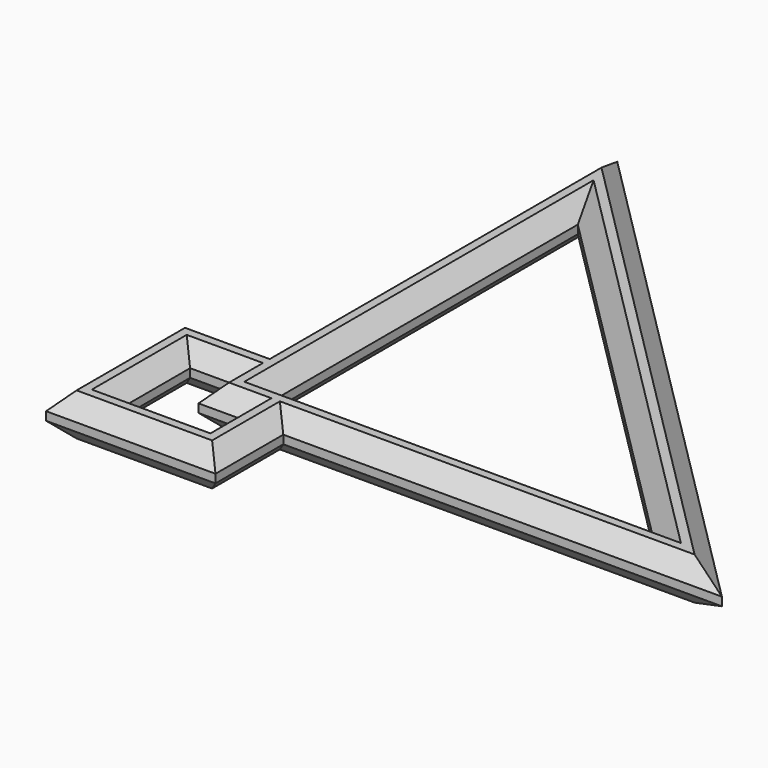
from build123d import *

# Parameters (mm, degrees)
F1_DEPTH      = 6.35
F2_T1_DEPTH   = 59.4126841144
F2_T3_DEPTH   = 12.7
F2_T5_DEPTH   = 25.4
F2_T7_DEPTH   = 25.4
F2_T9_DEPTH   = 12.7
F2_T11_DEPTH  = 12.7
F2_T13_DEPTH  = 12.7
F2_T15_DEPTH  = 6.35
F2_T17_DEPTH  = 6.35
F2_T19_DEPTH  = 6.35
F2_T21_DEPTH  = 6.35
F2_T26_DEPTH  = 63.3145027828
F2_T31_DEPTH  = 93.3666293515
F2_T37_DEPTH  = 63.3145027828
F2_T42_DEPTH  = 72.2947589038
F2_T47_DEPTH  = 124.0271405833
F2_T53_DEPTH  = 12.882074075
F2_T58_DEPTH  = 63.3145027828
F2_T63_DEPTH  = 93.3666293515
F2_T69_DEPTH  = 63.3145027828
F2_T74_DEPTH  = 72.2947589038
F2_T79_DEPTH  = 124.0271405833
F2_T85_DEPTH  = 12.882074075
F2_T91_DEPTH  = 69.8465775722
F2_T95_DEPTH  = 69.8465775722
F2_T102_DEPTH = 63.3145027828
F2_T106_DEPTH = 93.3666293515
F2_T113_DEPTH = 93.3666293515
F2_T117_DEPTH = 63.3145027828
F2_T124_DEPTH = 65.9447589038
F2_T128_DEPTH = 19.2320747894
F2_T135_DEPTH = 19.2320747894
F2_T139_DEPTH = 31.9320747894
F2_T146_DEPTH = 31.9320747894
F2_T150_DEPTH = 31.9320747894
F2_T157_DEPTH = 31.9320747894
F2_T161_DEPTH = 19.2320747894
F2_T168_DEPTH = 19.2320747894
F2_T172_DEPTH = 78.8268336933
F2_T179_DEPTH = 72.2947589038
F2_T183_DEPTH = 124.0271405833
F2_T190_DEPTH = 124.0271405833
F2_T194_DEPTH = 12.882074075
F2_T201_DEPTH = 19.2320747894
F2_T205_DEPTH = 12.8820747894
F2_T212_DEPTH = 19.2320747894
F2_T216_DEPTH = 19.2320747894
F2_T223_DEPTH = 19.2320747894
F2_T227_DEPTH = 12.8820747894
F2_T234_DEPTH = 12.8820747894
F2_T238_DEPTH = 12.8820747894
F2_T245_DEPTH = 12.8820747894
F2_T249_DEPTH = 12.8820747894
F2_T256_DEPTH = 12.8820747894
F2_T260_DEPTH = 12.8820747894
F2_T267_DEPTH = 69.8465775722
F2_T271_DEPTH = 69.8465775722
F2_T278_DEPTH = 63.3145027828
F2_T282_DEPTH = 93.3666293515
F2_T289_DEPTH = 93.3666293515
F2_T293_DEPTH = 63.3145027828
F2_T300_DEPTH = 65.9447589038
F2_T304_DEPTH = 19.2320747894
F2_T311_DEPTH = 19.2320747894
F2_T315_DEPTH = 31.9320747894
F2_T322_DEPTH = 31.9320747894
F2_T326_DEPTH = 31.9320747894
F2_T333_DEPTH = 31.9320747894
F2_T337_DEPTH = 19.2320747894
F2_T344_DEPTH = 19.2320747894
F2_T348_DEPTH = 78.8268336933
F2_T355_DEPTH = 72.2947589038
F2_T359_DEPTH = 124.0271405833
F2_T366_DEPTH = 124.0271405833
F2_T370_DEPTH = 12.882074075
F2_T377_DEPTH = 19.2320747894
F2_T381_DEPTH = 12.8820747894
F2_T388_DEPTH = 19.2320747894
F2_T392_DEPTH = 19.2320747894
F2_T399_DEPTH = 19.2320747894
F2_T403_DEPTH = 12.8820747894
F2_T410_DEPTH = 12.8820747894
F2_T414_DEPTH = 12.8820747894
F2_T421_DEPTH = 12.8820747894
F2_T425_DEPTH = 12.8820747894
F2_T432_DEPTH = 12.8820747894
F2_T436_DEPTH = 12.8820747894


# Not quite as in the source:
# - a fillet or chamfer that OpenCascade refuses, or shapes differently, is made with other operations: its cross-section is extruded or revolved along the edge and cut away or added


with BuildPart() as f1:
    # F0 (on Top) → F1 (new body)
    with BuildSketch(Plane.XY):
        Polygon((3.3168498194, -3.4059576905), (62.7295339338, -3.4059576905), (62.7295339338, 2.9440423095), (53.7492778127, 2.9440423095), (-3.0331501806, 2.9440423095), (-3.0331501806, 59.7264703029), (-3.0331501806, 68.7067264239), (-9.3831501806, 68.7067264239), (-9.3831501806, 9.2940423095), (-22.0831501806, 9.2940423095), (-22.0831501806, -16.1059576905), (3.3168498194, -16.1059576905), align=None)
        Polygon((-15.7331501806, -9.7559576905), (-15.7331501806, 2.9440423095), (-9.3831501806, 2.9440423095), (-9.3831501806, -3.4059576905), (-3.0331501806, -3.4059576905), (-3.0331501806, -9.7559576905), align=None, mode=Mode.SUBTRACT)
        Polygon((53.7492778127, 2.9440423095), (62.7295339338, 2.9440423095), (-3.0331501806, 68.7067264239), (-3.0331501806, 59.7264703029), align=None)
        Polygon((-9.3831501806, 68.7067264239), (-3.0331501806, 68.7067264239), (-9.3831494662, 75.0567257095), (-9.3831497783, 72.282161946), align=None)
        Polygon((62.7295339338, 2.9440423095), (62.7295339338, -3.4059576905), (69.0795339338, -3.4059576905), align=None)
    extrude(amount=F1_DEPTH)

    # F2: chamfer of 2.54 on 34 edges, made by hand

    # F2_s2 → F2_t1 (cut)
    with BuildSketch(Plane.XZ.offset(-68.7067264239)):
        with BuildLine():
            Line((-9.4549922296, 3.738157951), (-6.7713081316, 6.421842049))
            Line((-6.7713081316, 6.421842049), (-6.7713081316, 6.472642049))
            ThreePointArc((-6.7713081316, 6.472642049), (-8.0772291561, 6.4008), (-9.3831501806, 6.4008))
            Line((-9.3831501806, 6.4008), (-9.4339501806, 6.35))
            ThreePointArc((-9.4339501806, 6.35), (-9.4339501806, 5.0440789755), (-9.5057922296, 3.738157951))
            Line((-9.5057922296, 3.738157951), (-9.4549922296, 3.738157951))
        make_face()
        with BuildLine():
            Line((-9.4549922296, 2.611842049), (-6.7713081316, -0.071842049))
            Line((-6.7713081316, -0.071842049), (-6.7713081316, -0.122642049))
            ThreePointArc((-6.7713081316, -0.122642049), (-8.0772291561, -0.0508), (-9.3831501806, -0.0508))
            Line((-9.3831501806, -0.0508), (-9.4339501806, 0))
            ThreePointArc((-9.4339501806, 0), (-9.4339501806, 1.3059210245), (-9.5057922296, 2.611842049))
            Line((-9.5057922296, 2.611842049), (-9.4549922296, 2.611842049))
        make_face()
    extrude(amount=F2_T1_DEPTH, mode=Mode.SUBTRACT)

    # F2_s4 → F2_t3 (cut)
    with BuildSketch(Plane.YZ.offset(-22.0831501806)):
        with BuildLine():
            Line((9.3658843585, 3.738157951), (6.6822002606, 6.421842049))
            Line((6.6822002606, 6.421842049), (6.6822002606, 6.472642049))
            ThreePointArc((6.6822002606, 6.472642049), (7.9881212851, 6.4008), (9.2940423095, 6.4008))
            Line((9.2940423095, 6.4008), (9.3448423095, 6.35))
            ThreePointArc((9.3448423095, 6.35), (9.3448423095, 5.0440789755), (9.4166843585, 3.738157951))
            Line((9.4166843585, 3.738157951), (9.3658843585, 3.738157951))
        make_face()
        with BuildLine():
            Line((9.3658843585, 2.611842049), (6.6822002606, -0.071842049))
            Line((6.6822002606, -0.071842049), (6.6822002606, -0.122642049))
            ThreePointArc((6.6822002606, -0.122642049), (7.9881212851, -0.0508), (9.2940423095, -0.0508))
            Line((9.2940423095, -0.0508), (9.3448423095, 0))
            ThreePointArc((9.3448423095, 0), (9.3448423095, 1.3059210245), (9.4166843585, 2.611842049))
            Line((9.4166843585, 2.611842049), (9.3658843585, 2.611842049))
        make_face()
    extrude(amount=F2_T3_DEPTH, mode=Mode.SUBTRACT)

    # F2_s6 → F2_t5 (cut)
    with BuildSketch(Plane.XZ.offset(-9.2940423095)):
        with BuildLine():
            Line((-22.1549922296, 3.738157951), (-19.4713081316, 6.421842049))
            Line((-19.4713081316, 6.421842049), (-19.4713081316, 6.472642049))
            ThreePointArc((-19.4713081316, 6.472642049), (-20.7772291561, 6.4008), (-22.0831501806, 6.4008))
            Line((-22.0831501806, 6.4008), (-22.1339501806, 6.35))
            ThreePointArc((-22.1339501806, 6.35), (-22.1339501806, 5.0440789755), (-22.2057922296, 3.738157951))
            Line((-22.2057922296, 3.738157951), (-22.1549922296, 3.738157951))
        make_face()
        with BuildLine():
            Line((-22.1549922296, 2.611842049), (-19.4713081316, -0.071842049))
            Line((-19.4713081316, -0.071842049), (-19.4713081316, -0.122642049))
            ThreePointArc((-19.4713081316, -0.122642049), (-20.7772291561, -0.0508), (-22.0831501806, -0.0508))
            Line((-22.0831501806, -0.0508), (-22.1339501806, 0))
            ThreePointArc((-22.1339501806, 0), (-22.1339501806, 1.3059210245), (-22.2057922296, 2.611842049))
            Line((-22.2057922296, 2.611842049), (-22.1549922296, 2.611842049))
        make_face()
    extrude(amount=F2_T5_DEPTH, mode=Mode.SUBTRACT)

    # F2_s8 → F2_t7 (cut)
    with BuildSketch(Plane.YZ.offset(-22.0831501806)):
        with BuildLine():
            Line((-16.1777997394, 3.738157951), (-13.4941156415, 6.421842049))
            Line((-13.4941156415, 6.421842049), (-13.4941156415, 6.472642049))
            ThreePointArc((-13.4941156415, 6.472642049), (-14.800036666, 6.4008), (-16.1059576905, 6.4008))
            Line((-16.1059576905, 6.4008), (-16.1567576905, 6.35))
            ThreePointArc((-16.1567576905, 6.35), (-16.1567576905, 5.0440789755), (-16.2285997394, 3.738157951))
            Line((-16.2285997394, 3.738157951), (-16.1777997394, 3.738157951))
        make_face()
        with BuildLine():
            Line((-16.1777997394, 2.611842049), (-13.4941156415, -0.071842049))
            Line((-13.4941156415, -0.071842049), (-13.4941156415, -0.122642049))
            ThreePointArc((-13.4941156415, -0.122642049), (-14.800036666, -0.0508), (-16.1059576905, -0.0508))
            Line((-16.1059576905, -0.0508), (-16.1567576905, 0))
            ThreePointArc((-16.1567576905, 0), (-16.1567576905, 1.3059210245), (-16.2285997394, 2.611842049))
            Line((-16.2285997394, 2.611842049), (-16.1777997394, 2.611842049))
        make_face()
    extrude(amount=F2_T7_DEPTH, mode=Mode.SUBTRACT)

    # F2_s10 → F2_t9 (cut)
    with BuildSketch(Plane.XZ.offset(3.4059576905)):
        with BuildLine():
            Line((3.3886918684, 3.738157951), (0.7050077704, 6.421842049))
            Line((0.7050077704, 6.421842049), (0.7050077704, 6.472642049))
            ThreePointArc((0.7050077704, 6.472642049), (2.0109287949, 6.4008), (3.3168498194, 6.4008))
            Line((3.3168498194, 6.4008), (3.3676498194, 6.35))
            ThreePointArc((3.3676498194, 6.35), (3.3676498194, 5.0440789755), (3.4394918684, 3.738157951))
            Line((3.4394918684, 3.738157951), (3.3886918684, 3.738157951))
        make_face()
        with BuildLine():
            Line((3.3886918684, 2.611842049), (0.7050077704, -0.071842049))
            Line((0.7050077704, -0.071842049), (0.7050077704, -0.122642049))
            ThreePointArc((0.7050077704, -0.122642049), (2.0109287949, -0.0508), (3.3168498194, -0.0508))
            Line((3.3168498194, -0.0508), (3.3676498194, 0))
            ThreePointArc((3.3676498194, 0), (3.3676498194, 1.3059210245), (3.4394918684, 2.611842049))
            Line((3.4394918684, 2.611842049), (3.3886918684, 2.611842049))
        make_face()
    extrude(amount=F2_T9_DEPTH, mode=Mode.SUBTRACT)

    # F2_s12 → F2_t11 (cut)
    with BuildSketch(Plane.YZ.offset(-15.7331501806)):
        with BuildLine():
            Line((-9.6841156415, 3.738157951), (-12.3677997394, 6.421842049))
            Line((-12.3677997394, 6.421842049), (-12.3677997394, 6.472642049))
            ThreePointArc((-12.3677997394, 6.472642049), (-11.0618787149, 6.4008), (-9.7559576905, 6.4008))
            Line((-9.7559576905, 6.4008), (-9.7051576905, 6.35))
            ThreePointArc((-9.7051576905, 6.35), (-9.7051576905, 5.0440789755), (-9.6333156415, 3.738157951))
            Line((-9.6333156415, 3.738157951), (-9.6841156415, 3.738157951))
        make_face()
        with BuildLine():
            Line((-9.6841156415, 2.611842049), (-12.3677997394, -0.071842049))
            Line((-12.3677997394, -0.071842049), (-12.3677997394, -0.122642049))
            ThreePointArc((-12.3677997394, -0.122642049), (-11.0618787149, -0.0508), (-9.7559576905, -0.0508))
            Line((-9.7559576905, -0.0508), (-9.7051576905, 0))
            ThreePointArc((-9.7051576905, 0), (-9.7051576905, 1.3059210245), (-9.6333156415, 2.611842049))
            Line((-9.6333156415, 2.611842049), (-9.6841156415, 2.611842049))
        make_face()
    extrude(amount=F2_T11_DEPTH, mode=Mode.SUBTRACT)

    # F2_s14 → F2_t13 (cut)
    with BuildSketch(Plane.XZ.offset(-2.9440423095)):
        with BuildLine():
            Line((-15.6613081316, 3.738157951), (-18.3449922296, 6.421842049))
            Line((-18.3449922296, 6.421842049), (-18.3449922296, 6.472642049))
            ThreePointArc((-18.3449922296, 6.472642049), (-17.0390712051, 6.4008), (-15.7331501806, 6.4008))
            Line((-15.7331501806, 6.4008), (-15.6823501806, 6.35))
            ThreePointArc((-15.6823501806, 6.35), (-15.6823501806, 5.0440789755), (-15.6105081316, 3.738157951))
            Line((-15.6105081316, 3.738157951), (-15.6613081316, 3.738157951))
        make_face()
        with BuildLine():
            Line((-15.6613081316, 2.611842049), (-18.3449922296, -0.071842049))
            Line((-18.3449922296, -0.071842049), (-18.3449922296, -0.122642049))
            ThreePointArc((-18.3449922296, -0.122642049), (-17.0390712051, -0.0508), (-15.7331501806, -0.0508))
            Line((-15.7331501806, -0.0508), (-15.6823501806, 0))
            ThreePointArc((-15.6823501806, 0), (-15.6823501806, 1.3059210245), (-15.6105081316, 2.611842049))
            Line((-15.6105081316, 2.611842049), (-15.6613081316, 2.611842049))
        make_face()
    extrude(amount=F2_T13_DEPTH, mode=Mode.SUBTRACT)

    # F2_s16 → F2_t15 (cut)
    with BuildSketch(Plane.YZ.offset(-15.7331501806)):
        with BuildLine():
            Line((2.8722002606, 3.738157951), (5.5558843585, 6.421842049))
            Line((5.5558843585, 6.421842049), (5.5558843585, 6.472642049))
            ThreePointArc((5.5558843585, 6.472642049), (4.249963334, 6.4008), (2.9440423095, 6.4008))
            Line((2.9440423095, 6.4008), (2.8932423095, 6.35))
            ThreePointArc((2.8932423095, 6.35), (2.8932423095, 5.0440789755), (2.8214002606, 3.738157951))
            Line((2.8214002606, 3.738157951), (2.8722002606, 3.738157951))
        make_face()
        with BuildLine():
            Line((2.8722002606, 2.611842049), (5.5558843585, -0.071842049))
            Line((5.5558843585, -0.071842049), (5.5558843585, -0.122642049))
            ThreePointArc((5.5558843585, -0.122642049), (4.249963334, -0.0508), (2.9440423095, -0.0508))
            Line((2.9440423095, -0.0508), (2.8932423095, 0))
            ThreePointArc((2.8932423095, 0), (2.8932423095, 1.3059210245), (2.8214002606, 2.611842049))
            Line((2.8214002606, 2.611842049), (2.8722002606, 2.611842049))
        make_face()
    extrude(amount=F2_T15_DEPTH, mode=Mode.SUBTRACT)

    # F2_s18 → F2_t17 (cut)
    with BuildSketch(Plane.XZ.offset(-2.9440423095)):
        with BuildLine():
            Line((-9.4549922296, 3.738157951), (-6.7713081316, 6.421842049))
            Line((-6.7713081316, 6.421842049), (-6.7713081316, 6.472642049))
            ThreePointArc((-6.7713081316, 6.472642049), (-8.0772291561, 6.4008), (-9.3831501806, 6.4008))
            Line((-9.3831501806, 6.4008), (-9.4339501806, 6.35))
            ThreePointArc((-9.4339501806, 6.35), (-9.4339501806, 5.0440789755), (-9.5057922296, 3.738157951))
            Line((-9.5057922296, 3.738157951), (-9.4549922296, 3.738157951))
        make_face()
        with BuildLine():
            Line((-9.4549922296, 2.611842049), (-6.7713081316, -0.071842049))
            Line((-6.7713081316, -0.071842049), (-6.7713081316, -0.122642049))
            ThreePointArc((-6.7713081316, -0.122642049), (-8.0772291561, -0.0508), (-9.3831501806, -0.0508))
            Line((-9.3831501806, -0.0508), (-9.4339501806, 0))
            ThreePointArc((-9.4339501806, 0), (-9.4339501806, 1.3059210245), (-9.5057922296, 2.611842049))
            Line((-9.5057922296, 2.611842049), (-9.4549922296, 2.611842049))
        make_face()
    extrude(amount=F2_T17_DEPTH, mode=Mode.SUBTRACT)

    # F2_s20 → F2_t19 (cut)
    with BuildSketch(Plane.YZ.offset(-9.3831501806)):
        with BuildLine():
            Line((-3.4777997394, 3.738157951), (-0.7941156415, 6.421842049))
            Line((-0.7941156415, 6.421842049), (-0.7941156415, 6.472642049))
            ThreePointArc((-0.7941156415, 6.472642049), (-2.100036666, 6.4008), (-3.4059576905, 6.4008))
            Line((-3.4059576905, 6.4008), (-3.4567576905, 6.35))
            ThreePointArc((-3.4567576905, 6.35), (-3.4567576905, 5.0440789755), (-3.5285997394, 3.738157951))
            Line((-3.5285997394, 3.738157951), (-3.4777997394, 3.738157951))
        make_face()
        with BuildLine():
            Line((-3.4777997394, 2.611842049), (-0.7941156415, -0.071842049))
            Line((-0.7941156415, -0.071842049), (-0.7941156415, -0.122642049))
            ThreePointArc((-0.7941156415, -0.122642049), (-2.100036666, -0.0508), (-3.4059576905, -0.0508))
            Line((-3.4059576905, -0.0508), (-3.4567576905, 0))
            ThreePointArc((-3.4567576905, 0), (-3.4567576905, 1.3059210245), (-3.5285997394, 2.611842049))
            Line((-3.5285997394, 2.611842049), (-3.4777997394, 2.611842049))
        make_face()
    extrude(amount=F2_T19_DEPTH, mode=Mode.SUBTRACT)

    # F2_s22 → F2_t21 (cut)
    with BuildSketch(Plane.XZ.offset(3.4059576905)):
        with BuildLine():
            Line((-3.1049922296, 3.738157951), (-0.4213081316, 6.421842049))
            Line((-0.4213081316, 6.421842049), (-0.4213081316, 6.472642049))
            ThreePointArc((-0.4213081316, 6.472642049), (-1.7272291561, 6.4008), (-3.0331501806, 6.4008))
            Line((-3.0331501806, 6.4008), (-3.0839501806, 6.35))
            ThreePointArc((-3.0839501806, 6.35), (-3.0839501806, 5.0440789755), (-3.1557922296, 3.738157951))
            Line((-3.1557922296, 3.738157951), (-3.1049922296, 3.738157951))
        make_face()
        with BuildLine():
            Line((-3.1049922296, 2.611842049), (-0.4213081316, -0.071842049))
            Line((-0.4213081316, -0.071842049), (-0.4213081316, -0.122642049))
            ThreePointArc((-0.4213081316, -0.122642049), (-1.7272291561, -0.0508), (-3.0331501806, -0.0508))
            Line((-3.0331501806, -0.0508), (-3.0839501806, 0))
            ThreePointArc((-3.0839501806, 0), (-3.0839501806, 1.3059210245), (-3.1557922296, 2.611842049))
            Line((-3.1557922296, 2.611842049), (-3.1049922296, 2.611842049))
        make_face()
    extrude(amount=F2_T21_DEPTH, mode=Mode.SUBTRACT)


with BuildPart() as f2_tool24:
    # F2_s25 → F2_t26 (new body)
    with BuildSketch(Plane.XZ.offset(-2.9440423095)):
        with BuildLine():
            Line((-2.9613081316, 3.738157951), (-5.6449922296, 6.421842049))
            Line((-5.6449922296, 6.421842049), (-5.6449922296, 6.472642049))
            ThreePointArc((-5.6449922296, 6.472642049), (-4.3390712051, 6.4008), (-3.0331501806, 6.4008))
            Line((-3.0331501806, 6.4008), (-2.9823501806, 6.35))
            ThreePointArc((-2.9823501806, 6.35), (-2.9823501806, 5.0440789755), (-2.9105081316, 3.738157951))
            Line((-2.9105081316, 3.738157951), (-2.9613081316, 3.738157951))
        make_face()
    extrude(amount=-F2_T26_DEPTH)

    split(bisect_by=Plane(origin=(28.3466600611, 28.3466600611, 0), x_dir=(0, 0, 1), z_dir=(-0.7071067812, -0.7071067812, 0)), keep=Keep.TOP)


with BuildPart() as f1_1:
    add(f1.part)

    # F2_t23: cut F2_tool24
    add(f2_tool24.part, mode=Mode.SUBTRACT)


with BuildPart() as f2_tool29:
    # F2_s30 → F2_t31 (new body)
    with BuildSketch(Plane(origin=(-35.9986846206, 35.9986846206, 0), x_dir=(0, 0, 1), z_dir=(0.7071067812, -0.7071067812, 0))):
        with BuildLine():
            Line((3.738157951, -40.0163890575), (6.421842049, -42.7000731554))
            Line((6.421842049, -42.7000731554), (6.472642049, -42.7000731554))
            ThreePointArc((6.472642049, -42.7000731554), (6.4008, -41.3941521309), (6.4008, -40.0882311064))
            Line((6.4008, -40.0882311064), (6.35, -40.0374311064))
            ThreePointArc((6.35, -40.0374311064), (5.0440789755, -40.0374311064), (3.738157951, -39.9655890575))
            Line((3.738157951, -39.9655890575), (3.738157951, -40.0163890575))
        make_face()
    extrude(amount=F2_T31_DEPTH)

    split(bisect_by=Plane.YZ.offset(-3.0331501806), keep=Keep.TOP)

    split(bisect_by=Plane.XZ.offset(-2.9440423095), keep=Keep.BOTTOM)


with BuildPart() as f1_2:
    add(f1_1.part)

    # F2_t28: cut F2_tool29
    add(f2_tool29.part, mode=Mode.SUBTRACT)


with BuildPart() as f2_tool35:
    # F2_s36 → F2_t37 (new body)
    with BuildSketch(Plane.YZ.offset(60.2813526022)):
        with BuildLine():
            Line((3.0158843585, 3.738157951), (0.3322002606, 6.421842049))
            Line((0.3322002606, 6.421842049), (0.3322002606, 6.472642049))
            ThreePointArc((0.3322002606, 6.472642049), (1.6381212851, 6.4008), (2.9440423095, 6.4008))
            Line((2.9440423095, 6.4008), (2.9948423095, 6.35))
            ThreePointArc((2.9948423095, 6.35), (2.9948423095, 5.0440789755), (3.0666843585, 3.738157951))
            Line((3.0666843585, 3.738157951), (3.0158843585, 3.738157951))
        make_face()
    extrude(amount=-F2_T37_DEPTH)

    split(bisect_by=Plane(origin=(28.3466600611, 28.3466600611, 0), x_dir=(0, 0, 1), z_dir=(-0.7071067812, -0.7071067812, 0)), keep=Keep.TOP)


with BuildPart() as f1_3:
    add(f1_2.part)

    # F2_t34: cut F2_tool35
    add(f2_tool35.part, mode=Mode.SUBTRACT)


with BuildPart() as f2_tool40:
    # F2_s41 → F2_t42 (new body)
    with BuildSketch(Plane.YZ.offset(3.3168498194)):
        with BuildLine():
            Line((-3.4777997394, 3.738157951), (-0.7941156415, 6.421842049))
            Line((-0.7941156415, 6.421842049), (-0.7941156415, 6.472642049))
            ThreePointArc((-0.7941156415, 6.472642049), (-2.100036666, 6.4008), (-3.4059576905, 6.4008))
            Line((-3.4059576905, 6.4008), (-3.4567576905, 6.35))
            ThreePointArc((-3.4567576905, 6.35), (-3.4567576905, 5.0440789755), (-3.5285997394, 3.738157951))
            Line((-3.5285997394, 3.738157951), (-3.4777997394, 3.738157951))
        make_face()
    extrude(amount=F2_T42_DEPTH)

    split(bisect_by=Plane(origin=(32.8367881217, 32.8367881217, 0), x_dir=(0, 0, 1), z_dir=(-0.7071067812, -0.7071067812, 0)), keep=Keep.TOP)


with BuildPart() as f1_4:
    add(f1_3.part)

    # F2_t39: cut F2_tool40
    add(f2_tool40.part, mode=Mode.SUBTRACT)


with BuildPart() as f2_tool45:
    # F2_s46 → F2_t47 (new body)
    with BuildSketch(Plane(origin=(40.861620191, -40.861620191, 0), x_dir=(0, 0, 1), z_dir=(-0.7071067812, 0.7071067812, 0))):
        with BuildLine():
            Line((3.738157951, 46.5100731554), (6.421842049, 43.8263890575))
            Line((6.421842049, 43.8263890575), (6.472642049, 43.8263890575))
            ThreePointArc((6.472642049, 43.8263890575), (6.4008, 45.1323100819), (6.4008, 46.4382311064))
            Line((6.4008, 46.4382311064), (6.35, 46.4890311064))
            ThreePointArc((6.35, 46.4890311064), (5.0440789755, 46.4890311064), (3.738157951, 46.5608731554))
            Line((3.738157951, 46.5608731554), (3.738157951, 46.5100731554))
        make_face()
    extrude(amount=F2_T47_DEPTH)

    split(bisect_by=Plane.XZ.offset(3.4059576905), keep=Keep.BOTTOM)

    split(bisect_by=Plane.YZ.offset(-9.3831588139), keep=Keep.TOP)


with BuildPart() as f1_5:
    add(f1_4.part)

    # F2_t44: cut F2_tool45
    add(f2_tool45.part, mode=Mode.SUBTRACT)


with BuildPart() as f2_tool51:
    # F2_s52 → F2_t53 (new body)
    with BuildSketch(Plane.XZ.offset(-81.5888004989)):
        with BuildLine():
            Line((-9.4549907802, 3.738157951), (-6.7713066822, 6.421842049))
            Line((-6.7713066822, 6.421842049), (-6.7713066822, 6.472642049))
            ThreePointArc((-6.7713066822, 6.472642049), (-8.0772277067, 6.4008), (-9.3831487312, 6.4008))
            Line((-9.3831487312, 6.4008), (-9.4339487312, 6.35))
            ThreePointArc((-9.4339487312, 6.35), (-9.4339487312, 5.0440789755), (-9.5057907802, 3.738157951))
            Line((-9.5057907802, 3.738157951), (-9.4549907802, 3.738157951))
        make_face()
    extrude(amount=F2_T53_DEPTH)

    split(bisect_by=Plane(origin=(32.8367881217, 32.8367881217, 0), x_dir=(0, 0, 1), z_dir=(-0.7071067812, -0.7071067812, 0)), keep=Keep.TOP)


with BuildPart() as f1_6:
    add(f1_5.part)

    # F2_t50: cut F2_tool51
    add(f2_tool51.part, mode=Mode.SUBTRACT)


with BuildPart() as f2_tool56:
    # F2_s57 → F2_t58 (new body)
    with BuildSketch(Plane.XZ.offset(-2.9440423095)):
        with BuildLine():
            Line((-2.9613081316, 2.611842049), (-5.6449922296, -0.071842049))
            Line((-5.6449922296, -0.071842049), (-5.6449922296, -0.122642049))
            ThreePointArc((-5.6449922296, -0.122642049), (-4.3390712051, -0.0508), (-3.0331501806, -0.0508))
            Line((-3.0331501806, -0.0508), (-2.9823501806, 0))
            ThreePointArc((-2.9823501806, 0), (-2.9823501806, 1.3059210245), (-2.9105081316, 2.611842049))
            Line((-2.9105081316, 2.611842049), (-2.9613081316, 2.611842049))
        make_face()
    extrude(amount=-F2_T58_DEPTH)

    split(bisect_by=Plane(origin=(28.3466600611, 28.3466600611, 0), x_dir=(0, 0, 1), z_dir=(-0.7071067812, -0.7071067812, 0)), keep=Keep.TOP)


with BuildPart() as f1_7:
    add(f1_6.part)

    # F2_t55: cut F2_tool56
    add(f2_tool56.part, mode=Mode.SUBTRACT)


with BuildPart() as f2_tool61:
    # F2_s62 → F2_t63 (new body)
    with BuildSketch(Plane(origin=(-35.9986846206, 35.9986846206, 0), x_dir=(0, 0, 1), z_dir=(0.7071067812, -0.7071067812, 0))):
        with BuildLine():
            Line((2.611842049, -40.0163890575), (-0.071842049, -42.7000731554))
            Line((-0.071842049, -42.7000731554), (-0.122642049, -42.7000731554))
            ThreePointArc((-0.122642049, -42.7000731554), (-0.0508, -41.3941521309), (-0.0508, -40.0882311064))
            Line((-0.0508, -40.0882311064), (0, -40.0374311064))
            ThreePointArc((0, -40.0374311064), (1.3059210245, -40.0374311064), (2.611842049, -39.9655890575))
            Line((2.611842049, -39.9655890575), (2.611842049, -40.0163890575))
        make_face()
    extrude(amount=F2_T63_DEPTH)

    split(bisect_by=Plane.YZ.offset(-3.0331501806), keep=Keep.TOP)

    split(bisect_by=Plane.XZ.offset(-2.9440423095), keep=Keep.BOTTOM)


with BuildPart() as f1_8:
    add(f1_7.part)

    # F2_t60: cut F2_tool61
    add(f2_tool61.part, mode=Mode.SUBTRACT)


with BuildPart() as f2_tool67:
    # F2_s68 → F2_t69 (new body)
    with BuildSketch(Plane.YZ.offset(60.2813526022)):
        with BuildLine():
            Line((3.0158843585, 2.611842049), (0.3322002606, -0.071842049))
            Line((0.3322002606, -0.071842049), (0.3322002606, -0.122642049))
            ThreePointArc((0.3322002606, -0.122642049), (1.6381212851, -0.0508), (2.9440423095, -0.0508))
            Line((2.9440423095, -0.0508), (2.9948423095, 0))
            ThreePointArc((2.9948423095, 0), (2.9948423095, 1.3059210245), (3.0666843585, 2.611842049))
            Line((3.0666843585, 2.611842049), (3.0158843585, 2.611842049))
        make_face()
    extrude(amount=-F2_T69_DEPTH)

    split(bisect_by=Plane(origin=(28.3466600611, 28.3466600611, 0), x_dir=(0, 0, 1), z_dir=(-0.7071067812, -0.7071067812, 0)), keep=Keep.TOP)


with BuildPart() as f1_9:
    add(f1_8.part)

    # F2_t66: cut F2_tool67
    add(f2_tool67.part, mode=Mode.SUBTRACT)


with BuildPart() as f2_tool72:
    # F2_s73 → F2_t74 (new body)
    with BuildSketch(Plane.YZ.offset(3.3168498194)):
        with BuildLine():
            Line((-3.4777997394, 2.611842049), (-0.7941156415, -0.071842049))
            Line((-0.7941156415, -0.071842049), (-0.7941156415, -0.122642049))
            ThreePointArc((-0.7941156415, -0.122642049), (-2.100036666, -0.0508), (-3.4059576905, -0.0508))
            Line((-3.4059576905, -0.0508), (-3.4567576905, 0))
            ThreePointArc((-3.4567576905, 0), (-3.4567576905, 1.3059210245), (-3.5285997394, 2.611842049))
            Line((-3.5285997394, 2.611842049), (-3.4777997394, 2.611842049))
        make_face()
    extrude(amount=F2_T74_DEPTH)

    split(bisect_by=Plane(origin=(32.8367881217, 32.8367881217, 0), x_dir=(0, 0, 1), z_dir=(-0.7071067812, -0.7071067812, 0)), keep=Keep.TOP)


with BuildPart() as f1_10:
    add(f1_9.part)

    # F2_t71: cut F2_tool72
    add(f2_tool72.part, mode=Mode.SUBTRACT)


with BuildPart() as f2_tool77:
    # F2_s78 → F2_t79 (new body)
    with BuildSketch(Plane(origin=(40.861620191, -40.861620191, 0), x_dir=(0, 0, 1), z_dir=(-0.7071067812, 0.7071067812, 0))):
        with BuildLine():
            Line((2.611842049, 46.5100731554), (-0.071842049, 43.8263890575))
            Line((-0.071842049, 43.8263890575), (-0.122642049, 43.8263890575))
            ThreePointArc((-0.122642049, 43.8263890575), (-0.0508, 45.1323100819), (-0.0508, 46.4382311064))
            Line((-0.0508, 46.4382311064), (0, 46.4890311064))
            ThreePointArc((0, 46.4890311064), (1.3059210245, 46.4890311064), (2.611842049, 46.5608731554))
            Line((2.611842049, 46.5608731554), (2.611842049, 46.5100731554))
        make_face()
    extrude(amount=F2_T79_DEPTH)

    split(bisect_by=Plane.XZ.offset(3.4059576905), keep=Keep.BOTTOM)

    split(bisect_by=Plane.YZ.offset(-9.3831588139), keep=Keep.TOP)


with BuildPart() as f1_11:
    add(f1_10.part)

    # F2_t76: cut F2_tool77
    add(f2_tool77.part, mode=Mode.SUBTRACT)


with BuildPart() as f2_tool83:
    # F2_s84 → F2_t85 (new body)
    with BuildSketch(Plane.XZ.offset(-81.5888004989)):
        with BuildLine():
            Line((-9.4549907802, 2.611842049), (-6.7713066822, -0.071842049))
            Line((-6.7713066822, -0.071842049), (-6.7713066822, -0.122642049))
            ThreePointArc((-6.7713066822, -0.122642049), (-8.0772277067, -0.0508), (-9.3831487312, -0.0508))
            Line((-9.3831487312, -0.0508), (-9.4339487312, 0))
            ThreePointArc((-9.4339487312, 0), (-9.4339487312, 1.3059210245), (-9.5057907802, 2.611842049))
            Line((-9.5057907802, 2.611842049), (-9.4549907802, 2.611842049))
        make_face()
    extrude(amount=F2_T85_DEPTH)

    split(bisect_by=Plane(origin=(32.8367881217, 32.8367881217, 0), x_dir=(0, 0, 1), z_dir=(-0.7071067812, -0.7071067812, 0)), keep=Keep.TOP)


with BuildPart() as f1_12:
    add(f1_11.part)

    # F2_t82: cut F2_tool83
    add(f2_tool83.part, mode=Mode.SUBTRACT)


with BuildPart() as f2_tool89:
    # F2_s90 → F2_t91 (new body)
    with BuildSketch(Plane.XZ.offset(3.5880324799)):
        with BuildLine():
            Line((-2.9613081316, 3.738157951), (-5.6449922296, 6.421842049))
            Line((-5.6449922296, 6.421842049), (-5.6449922296, 6.472642049))
            ThreePointArc((-5.6449922296, 6.472642049), (-4.3390712051, 6.4008), (-3.0331501806, 6.4008))
            Line((-3.0331501806, 6.4008), (-2.9823501806, 6.35))
            ThreePointArc((-2.9823501806, 6.35), (-2.9823501806, 5.0440789755), (-2.9105081316, 3.738157951))
            Line((-2.9105081316, 3.738157951), (-2.9613081316, 3.738157951))
        make_face()
    extrude(amount=-F2_T91_DEPTH)

    split(bisect_by=Plane.XZ.offset(-2.9440423095), keep=Keep.TOP)


with BuildPart() as f2_tool93:
    # F2_s94 → F2_t95 (new body)
    with BuildSketch(Plane.YZ.offset(60.2813526022)):
        with BuildLine():
            Line((3.0158843585, 3.738157951), (0.3322002606, 6.421842049))
            Line((0.3322002606, 6.421842049), (0.3322002606, 6.472642049))
            ThreePointArc((0.3322002606, 6.472642049), (1.6381212851, 6.4008), (2.9440423095, 6.4008))
            Line((2.9440423095, 6.4008), (2.9948423095, 6.35))
            ThreePointArc((2.9948423095, 6.35), (2.9948423095, 5.0440789755), (3.0666843585, 3.738157951))
            Line((3.0666843585, 3.738157951), (3.0158843585, 3.738157951))
        make_face()
    extrude(amount=-F2_T95_DEPTH)

    split(bisect_by=Plane.YZ.offset(-3.0331501806), keep=Keep.BOTTOM)


with BuildPart() as f2_tool89_1:
    add(f2_tool89.part)

    # F2_t97: intersect F2_tool93
    add(f2_tool93.part, mode=Mode.INTERSECT)


with BuildPart() as f1_13:
    add(f1_12.part)

    # F2_t87: cut F2_tool89
    add(f2_tool89_1.part, mode=Mode.SUBTRACT)


with BuildPart() as f2_tool100:
    # F2_s101 → F2_t102 (new body)
    with BuildSketch(Plane.XZ.offset(-2.9440423095)):
        with BuildLine():
            Line((-2.9613081316, 3.738157951), (-5.6449922296, 6.421842049))
            Line((-5.6449922296, 6.421842049), (-5.6449922296, 6.472642049))
            ThreePointArc((-5.6449922296, 6.472642049), (-4.3390712051, 6.4008), (-3.0331501806, 6.4008))
            Line((-3.0331501806, 6.4008), (-2.9823501806, 6.35))
            ThreePointArc((-2.9823501806, 6.35), (-2.9823501806, 5.0440789755), (-2.9105081316, 3.738157951))
            Line((-2.9105081316, 3.738157951), (-2.9613081316, 3.738157951))
        make_face()
    extrude(amount=-F2_T102_DEPTH)

    split(bisect_by=Plane(origin=(28.3466600611, 28.3466600611, 0), x_dir=(0, 0, 1), z_dir=(0.7071067812, 0.7071067812, 0)), keep=Keep.TOP)


with BuildPart() as f2_tool104:
    # F2_s105 → F2_t106 (new body)
    with BuildSketch(Plane(origin=(-35.9986846206, 35.9986846206, 0), x_dir=(0, 0, 1), z_dir=(0.7071067812, -0.7071067812, 0))):
        with BuildLine():
            Line((3.738157951, -40.0163890575), (6.421842049, -42.7000731554))
            Line((6.421842049, -42.7000731554), (6.472642049, -42.7000731554))
            ThreePointArc((6.472642049, -42.7000731554), (6.4008, -41.3941521309), (6.4008, -40.0882311064))
            Line((6.4008, -40.0882311064), (6.35, -40.0374311064))
            ThreePointArc((6.35, -40.0374311064), (5.0440789755, -40.0374311064), (3.738157951, -39.9655890575))
            Line((3.738157951, -39.9655890575), (3.738157951, -40.0163890575))
        make_face()
    extrude(amount=F2_T106_DEPTH)

    split(bisect_by=Plane.YZ.offset(-3.0331501806), keep=Keep.BOTTOM)


with BuildPart() as f2_tool100_1:
    add(f2_tool100.part)

    # F2_t108: intersect F2_tool104
    add(f2_tool104.part, mode=Mode.INTERSECT)


with BuildPart() as f1_14:
    add(f1_13.part)

    # F2_t98: cut F2_tool100
    add(f2_tool100_1.part, mode=Mode.SUBTRACT)


with BuildPart() as f2_tool111:
    # F2_s112 → F2_t113 (new body)
    with BuildSketch(Plane(origin=(-35.9986846206, 35.9986846206, 0), x_dir=(0, 0, 1), z_dir=(0.7071067812, -0.7071067812, 0))):
        with BuildLine():
            Line((3.738157951, -40.0163890575), (6.421842049, -42.7000731554))
            Line((6.421842049, -42.7000731554), (6.472642049, -42.7000731554))
            ThreePointArc((6.472642049, -42.7000731554), (6.4008, -41.3941521309), (6.4008, -40.0882311064))
            Line((6.4008, -40.0882311064), (6.35, -40.0374311064))
            ThreePointArc((6.35, -40.0374311064), (5.0440789755, -40.0374311064), (3.738157951, -39.9655890575))
            Line((3.738157951, -39.9655890575), (3.738157951, -40.0163890575))
        make_face()
    extrude(amount=F2_T113_DEPTH)

    split(bisect_by=Plane.XZ.offset(-2.9440423095), keep=Keep.TOP)


with BuildPart() as f2_tool115:
    # F2_s116 → F2_t117 (new body)
    with BuildSketch(Plane.YZ.offset(60.2813526022)):
        with BuildLine():
            Line((3.0158843585, 3.738157951), (0.3322002606, 6.421842049))
            Line((0.3322002606, 6.421842049), (0.3322002606, 6.472642049))
            ThreePointArc((0.3322002606, 6.472642049), (1.6381212851, 6.4008), (2.9440423095, 6.4008))
            Line((2.9440423095, 6.4008), (2.9948423095, 6.35))
            ThreePointArc((2.9948423095, 6.35), (2.9948423095, 5.0440789755), (3.0666843585, 3.738157951))
            Line((3.0666843585, 3.738157951), (3.0158843585, 3.738157951))
        make_face()
    extrude(amount=-F2_T117_DEPTH)

    split(bisect_by=Plane(origin=(28.3466600611, 28.3466600611, 0), x_dir=(0, 0, 1), z_dir=(0.7071067812, 0.7071067812, 0)), keep=Keep.TOP)


with BuildPart() as f2_tool111_1:
    add(f2_tool111.part)

    # F2_t119: intersect F2_tool115
    add(f2_tool115.part, mode=Mode.INTERSECT)


with BuildPart() as f1_15:
    add(f1_14.part)

    # F2_t109: cut F2_tool111
    add(f2_tool111_1.part, mode=Mode.SUBTRACT)


with BuildPart() as f2_tool122:
    # F2_s123 → F2_t124 (new body)
    with BuildSketch(Plane.XZ.offset(-68.7067264239)):
        with BuildLine():
            Line((-9.4549922296, 3.738157951), (-6.7713081316, 6.421842049))
            Line((-6.7713081316, 6.421842049), (-6.7713081316, 6.472642049))
            ThreePointArc((-6.7713081316, 6.472642049), (-8.0772291561, 6.4008), (-9.3831501806, 6.4008))
            Line((-9.3831501806, 6.4008), (-9.4339501806, 6.35))
            ThreePointArc((-9.4339501806, 6.35), (-9.4339501806, 5.0440789755), (-9.5057922296, 3.738157951))
            Line((-9.5057922296, 3.738157951), (-9.4549922296, 3.738157951))
        make_face()
    extrude(amount=F2_T124_DEPTH)

    split(bisect_by=Plane.XZ.offset(-9.2940423095), keep=Keep.TOP)


with BuildPart() as f2_tool126:
    # F2_s127 → F2_t128 (new body)
    with BuildSketch(Plane.YZ.offset(-2.8510753912)):
        with BuildLine():
            Line((9.3658843585, 3.738157951), (6.6822002606, 6.421842049))
            Line((6.6822002606, 6.421842049), (6.6822002606, 6.472642049))
            ThreePointArc((6.6822002606, 6.472642049), (7.9881212851, 6.4008), (9.2940423095, 6.4008))
            Line((9.2940423095, 6.4008), (9.3448423095, 6.35))
            ThreePointArc((9.3448423095, 6.35), (9.3448423095, 5.0440789755), (9.4166843585, 3.738157951))
            Line((9.4166843585, 3.738157951), (9.3658843585, 3.738157951))
        make_face()
    extrude(amount=-F2_T128_DEPTH)

    split(bisect_by=Plane.YZ.offset(-9.3831501806), keep=Keep.TOP)


with BuildPart() as f2_tool122_1:
    add(f2_tool122.part)

    # F2_t130: intersect F2_tool126
    add(f2_tool126.part, mode=Mode.INTERSECT)


with BuildPart() as f1_16:
    add(f1_15.part)

    # F2_t120: cut F2_tool122
    add(f2_tool122_1.part, mode=Mode.SUBTRACT)


with BuildPart() as f2_tool133:
    # F2_s134 → F2_t135 (new body)
    with BuildSketch(Plane.YZ.offset(-9.3831501806)):
        with BuildLine():
            Line((9.3658843585, 3.738157951), (6.6822002606, 6.421842049))
            Line((6.6822002606, 6.421842049), (6.6822002606, 6.472642049))
            ThreePointArc((6.6822002606, 6.472642049), (7.9881212851, 6.4008), (9.2940423095, 6.4008))
            Line((9.2940423095, 6.4008), (9.3448423095, 6.35))
            ThreePointArc((9.3448423095, 6.35), (9.3448423095, 5.0440789755), (9.4166843585, 3.738157951))
            Line((9.4166843585, 3.738157951), (9.3658843585, 3.738157951))
        make_face()
    extrude(amount=-F2_T135_DEPTH)

    split(bisect_by=Plane.YZ.offset(-22.0831501806), keep=Keep.BOTTOM)


with BuildPart() as f2_tool137:
    # F2_s138 → F2_t139 (new body)
    with BuildSketch(Plane.XZ.offset(-15.826117099)):
        with BuildLine():
            Line((-22.1549922296, 3.738157951), (-19.4713081316, 6.421842049))
            Line((-19.4713081316, 6.421842049), (-19.4713081316, 6.472642049))
            ThreePointArc((-19.4713081316, 6.472642049), (-20.7772291561, 6.4008), (-22.0831501806, 6.4008))
            Line((-22.0831501806, 6.4008), (-22.1339501806, 6.35))
            ThreePointArc((-22.1339501806, 6.35), (-22.1339501806, 5.0440789755), (-22.2057922296, 3.738157951))
            Line((-22.2057922296, 3.738157951), (-22.1549922296, 3.738157951))
        make_face()
    extrude(amount=F2_T139_DEPTH)

    split(bisect_by=Plane.XZ.offset(-9.2940423095), keep=Keep.BOTTOM)


with BuildPart() as f2_tool133_1:
    add(f2_tool133.part)

    # F2_t141: intersect F2_tool137
    add(f2_tool137.part, mode=Mode.INTERSECT)


with BuildPart() as f1_17:
    add(f1_16.part)

    # F2_t131: cut F2_tool133
    add(f2_tool133_1.part, mode=Mode.SUBTRACT)


with BuildPart() as f2_tool144:
    # F2_s145 → F2_t146 (new body)
    with BuildSketch(Plane.XZ.offset(-9.2940423095)):
        with BuildLine():
            Line((-22.1549922296, 3.738157951), (-19.4713081316, 6.421842049))
            Line((-19.4713081316, 6.421842049), (-19.4713081316, 6.472642049))
            ThreePointArc((-19.4713081316, 6.472642049), (-20.7772291561, 6.4008), (-22.0831501806, 6.4008))
            Line((-22.0831501806, 6.4008), (-22.1339501806, 6.35))
            ThreePointArc((-22.1339501806, 6.35), (-22.1339501806, 5.0440789755), (-22.2057922296, 3.738157951))
            Line((-22.2057922296, 3.738157951), (-22.1549922296, 3.738157951))
        make_face()
    extrude(amount=F2_T146_DEPTH)

    split(bisect_by=Plane.XZ.offset(16.1059576905), keep=Keep.TOP)


with BuildPart() as f2_tool148:
    # F2_s149 → F2_t150 (new body)
    with BuildSketch(Plane.YZ.offset(-28.61522497)):
        with BuildLine():
            Line((-16.1777997394, 3.738157951), (-13.4941156415, 6.421842049))
            Line((-13.4941156415, 6.421842049), (-13.4941156415, 6.472642049))
            ThreePointArc((-13.4941156415, 6.472642049), (-14.800036666, 6.4008), (-16.1059576905, 6.4008))
            Line((-16.1059576905, 6.4008), (-16.1567576905, 6.35))
            ThreePointArc((-16.1567576905, 6.35), (-16.1567576905, 5.0440789755), (-16.2285997394, 3.738157951))
            Line((-16.2285997394, 3.738157951), (-16.1777997394, 3.738157951))
        make_face()
    extrude(amount=F2_T150_DEPTH)

    split(bisect_by=Plane.YZ.offset(-22.0831501806), keep=Keep.BOTTOM)


with BuildPart() as f2_tool144_1:
    add(f2_tool144.part)

    # F2_t152: intersect F2_tool148
    add(f2_tool148.part, mode=Mode.INTERSECT)


with BuildPart() as f1_18:
    add(f1_17.part)

    # F2_t142: cut F2_tool144
    add(f2_tool144_1.part, mode=Mode.SUBTRACT)


with BuildPart() as f2_tool155:
    # F2_s156 → F2_t157 (new body)
    with BuildSketch(Plane.YZ.offset(-22.0831501806)):
        with BuildLine():
            Line((-16.1777997394, 3.738157951), (-13.4941156415, 6.421842049))
            Line((-13.4941156415, 6.421842049), (-13.4941156415, 6.472642049))
            ThreePointArc((-13.4941156415, 6.472642049), (-14.800036666, 6.4008), (-16.1059576905, 6.4008))
            Line((-16.1059576905, 6.4008), (-16.1567576905, 6.35))
            ThreePointArc((-16.1567576905, 6.35), (-16.1567576905, 5.0440789755), (-16.2285997394, 3.738157951))
            Line((-16.2285997394, 3.738157951), (-16.1777997394, 3.738157951))
        make_face()
    extrude(amount=F2_T157_DEPTH)

    split(bisect_by=Plane.YZ.offset(3.3168498194), keep=Keep.TOP)


with BuildPart() as f2_tool159:
    # F2_s160 → F2_t161 (new body)
    with BuildSketch(Plane.XZ.offset(22.6380324799)):
        with BuildLine():
            Line((3.3886918684, 3.738157951), (0.7050077704, 6.421842049))
            Line((0.7050077704, 6.421842049), (0.7050077704, 6.472642049))
            ThreePointArc((0.7050077704, 6.472642049), (2.0109287949, 6.4008), (3.3168498194, 6.4008))
            Line((3.3168498194, 6.4008), (3.3676498194, 6.35))
            ThreePointArc((3.3676498194, 6.35), (3.3676498194, 5.0440789755), (3.4394918684, 3.738157951))
            Line((3.4394918684, 3.738157951), (3.3886918684, 3.738157951))
        make_face()
    extrude(amount=-F2_T161_DEPTH)

    split(bisect_by=Plane.XZ.offset(16.1059576905), keep=Keep.TOP)


with BuildPart() as f2_tool155_1:
    add(f2_tool155.part)

    # F2_t163: intersect F2_tool159
    add(f2_tool159.part, mode=Mode.INTERSECT)


with BuildPart() as f1_19:
    add(f1_18.part)

    # F2_t153: cut F2_tool155
    add(f2_tool155_1.part, mode=Mode.SUBTRACT)


with BuildPart() as f2_tool166:
    # F2_s167 → F2_t168 (new body)
    with BuildSketch(Plane.XZ.offset(16.1059576905)):
        with BuildLine():
            Line((3.3886918684, 3.738157951), (0.7050077704, 6.421842049))
            Line((0.7050077704, 6.421842049), (0.7050077704, 6.472642049))
            ThreePointArc((0.7050077704, 6.472642049), (2.0109287949, 6.4008), (3.3168498194, 6.4008))
            Line((3.3168498194, 6.4008), (3.3676498194, 6.35))
            ThreePointArc((3.3676498194, 6.35), (3.3676498194, 5.0440789755), (3.4394918684, 3.738157951))
            Line((3.4394918684, 3.738157951), (3.3886918684, 3.738157951))
        make_face()
    extrude(amount=-F2_T168_DEPTH)

    split(bisect_by=Plane.XZ.offset(3.4059576905), keep=Keep.BOTTOM)


with BuildPart() as f2_tool170:
    # F2_s171 → F2_t172 (new body)
    with BuildSketch(Plane.YZ.offset(-3.21522497)):
        with BuildLine():
            Line((-3.4777997394, 3.738157951), (-0.7941156415, 6.421842049))
            Line((-0.7941156415, 6.421842049), (-0.7941156415, 6.472642049))
            ThreePointArc((-0.7941156415, 6.472642049), (-2.100036666, 6.4008), (-3.4059576905, 6.4008))
            Line((-3.4059576905, 6.4008), (-3.4567576905, 6.35))
            ThreePointArc((-3.4567576905, 6.35), (-3.4567576905, 5.0440789755), (-3.5285997394, 3.738157951))
            Line((-3.5285997394, 3.738157951), (-3.4777997394, 3.738157951))
        make_face()
    extrude(amount=F2_T172_DEPTH)

    split(bisect_by=Plane.YZ.offset(3.3168498194), keep=Keep.BOTTOM)


with BuildPart() as f2_tool166_1:
    add(f2_tool166.part)

    # F2_t174: intersect F2_tool170
    add(f2_tool170.part, mode=Mode.INTERSECT)


with BuildPart() as f1_20:
    add(f1_19.part)

    # F2_t164: cut F2_tool166
    add(f2_tool166_1.part, mode=Mode.SUBTRACT)


with BuildPart() as f2_tool177:
    # F2_s178 → F2_t179 (new body)
    with BuildSketch(Plane.YZ.offset(3.3168498194)):
        with BuildLine():
            Line((-3.4777997394, 3.738157951), (-0.7941156415, 6.421842049))
            Line((-0.7941156415, 6.421842049), (-0.7941156415, 6.472642049))
            ThreePointArc((-0.7941156415, 6.472642049), (-2.100036666, 6.4008), (-3.4059576905, 6.4008))
            Line((-3.4059576905, 6.4008), (-3.4567576905, 6.35))
            ThreePointArc((-3.4567576905, 6.35), (-3.4567576905, 5.0440789755), (-3.5285997394, 3.738157951))
            Line((-3.5285997394, 3.738157951), (-3.4777997394, 3.738157951))
        make_face()
    extrude(amount=F2_T179_DEPTH)

    split(bisect_by=Plane(origin=(32.8367881217, 32.8367881217, 0), x_dir=(0, 0, 1), z_dir=(0.7071067812, 0.7071067812, 0)), keep=Keep.TOP)


with BuildPart() as f2_tool181:
    # F2_s182 → F2_t183 (new body)
    with BuildSketch(Plane(origin=(40.861620191, -40.861620191, 0), x_dir=(0, 0, 1), z_dir=(-0.7071067812, 0.7071067812, 0))):
        with BuildLine():
            Line((3.738157951, 46.5100731554), (6.421842049, 43.8263890575))
            Line((6.421842049, 43.8263890575), (6.472642049, 43.8263890575))
            ThreePointArc((6.472642049, 43.8263890575), (6.4008, 45.1323100819), (6.4008, 46.4382311064))
            Line((6.4008, 46.4382311064), (6.35, 46.4890311064))
            ThreePointArc((6.35, 46.4890311064), (5.0440789755, 46.4890311064), (3.738157951, 46.5608731554))
            Line((3.738157951, 46.5608731554), (3.738157951, 46.5100731554))
        make_face()
    extrude(amount=F2_T183_DEPTH)

    split(bisect_by=Plane.XZ.offset(3.4059576905), keep=Keep.TOP)


with BuildPart() as f2_tool177_1:
    add(f2_tool177.part)

    # F2_t185: intersect F2_tool181
    add(f2_tool181.part, mode=Mode.INTERSECT)


with BuildPart() as f1_21:
    add(f1_20.part)

    # F2_t175: cut F2_tool177
    add(f2_tool177_1.part, mode=Mode.SUBTRACT)


with BuildPart() as f2_tool188:
    # F2_s189 → F2_t190 (new body)
    with BuildSketch(Plane(origin=(40.861620191, -40.861620191, 0), x_dir=(0, 0, 1), z_dir=(-0.7071067812, 0.7071067812, 0))):
        with BuildLine():
            Line((3.738157951, 46.5100731554), (6.421842049, 43.8263890575))
            Line((6.421842049, 43.8263890575), (6.472642049, 43.8263890575))
            ThreePointArc((6.472642049, 43.8263890575), (6.4008, 45.1323100819), (6.4008, 46.4382311064))
            Line((6.4008, 46.4382311064), (6.35, 46.4890311064))
            ThreePointArc((6.35, 46.4890311064), (5.0440789755, 46.4890311064), (3.738157951, 46.5608731554))
            Line((3.738157951, 46.5608731554), (3.738157951, 46.5100731554))
        make_face()
    extrude(amount=F2_T190_DEPTH)

    split(bisect_by=Plane.YZ.offset(-9.3831588139), keep=Keep.BOTTOM)


with BuildPart() as f2_tool192:
    # F2_s193 → F2_t194 (new body)
    with BuildSketch(Plane.XZ.offset(-81.5888004989)):
        with BuildLine():
            Line((-9.4549907802, 3.738157951), (-6.7713066822, 6.421842049))
            Line((-6.7713066822, 6.421842049), (-6.7713066822, 6.472642049))
            ThreePointArc((-6.7713066822, 6.472642049), (-8.0772277067, 6.4008), (-9.3831487312, 6.4008))
            Line((-9.3831487312, 6.4008), (-9.4339487312, 6.35))
            ThreePointArc((-9.4339487312, 6.35), (-9.4339487312, 5.0440789755), (-9.5057907802, 3.738157951))
            Line((-9.5057907802, 3.738157951), (-9.4549907802, 3.738157951))
        make_face()
    extrude(amount=F2_T194_DEPTH)

    split(bisect_by=Plane(origin=(32.8367881217, 32.8367881217, 0), x_dir=(0, 0, 1), z_dir=(0.7071067812, 0.7071067812, 0)), keep=Keep.TOP)


with BuildPart() as f2_tool188_1:
    add(f2_tool188.part)

    # F2_t196: intersect F2_tool192
    add(f2_tool192.part, mode=Mode.INTERSECT)


with BuildPart() as f1_22:
    add(f1_21.part)

    # F2_t186: cut F2_tool188
    add(f2_tool188_1.part, mode=Mode.SUBTRACT)


with BuildPart() as f2_tool199:
    # F2_s200 → F2_t201 (new body)
    with BuildSketch(Plane.YZ.offset(3.4989246088)):
        with BuildLine():
            Line((-9.6841156415, 3.738157951), (-12.3677997394, 6.421842049))
            Line((-12.3677997394, 6.421842049), (-12.3677997394, 6.472642049))
            ThreePointArc((-12.3677997394, 6.472642049), (-11.0618787149, 6.4008), (-9.7559576905, 6.4008))
            Line((-9.7559576905, 6.4008), (-9.7051576905, 6.35))
            ThreePointArc((-9.7051576905, 6.35), (-9.7051576905, 5.0440789755), (-9.6333156415, 3.738157951))
            Line((-9.6333156415, 3.738157951), (-9.6841156415, 3.738157951))
        make_face()
    extrude(amount=-F2_T201_DEPTH)

    split(bisect_by=Plane.YZ.offset(-3.0331501806), keep=Keep.TOP)


with BuildPart() as f2_tool203:
    # F2_s204 → F2_t205 (new body)
    with BuildSketch(Plane.XZ.offset(3.4059576905)):
        with BuildLine():
            Line((-3.1049922296, 3.738157951), (-0.4213081316, 6.421842049))
            Line((-0.4213081316, 6.421842049), (-0.4213081316, 6.472642049))
            ThreePointArc((-0.4213081316, 6.472642049), (-1.7272291561, 6.4008), (-3.0331501806, 6.4008))
            Line((-3.0331501806, 6.4008), (-3.0839501806, 6.35))
            ThreePointArc((-3.0839501806, 6.35), (-3.0839501806, 5.0440789755), (-3.1557922296, 3.738157951))
            Line((-3.1557922296, 3.738157951), (-3.1049922296, 3.738157951))
        make_face()
    extrude(amount=F2_T205_DEPTH)

    split(bisect_by=Plane.XZ.offset(9.7559576905), keep=Keep.TOP)


with BuildPart() as f2_tool199_1:
    add(f2_tool199.part)

    # F2_t207: intersect F2_tool203
    add(f2_tool203.part, mode=Mode.INTERSECT)


with BuildPart() as f1_23:
    add(f1_22.part)

    # F2_t197: cut F2_tool199
    add(f2_tool199_1.part, mode=Mode.SUBTRACT)


with BuildPart() as f2_tool210:
    # F2_s211 → F2_t212 (new body)
    with BuildSketch(Plane.YZ.offset(-3.0331501806)):
        with BuildLine():
            Line((-9.6841156415, 3.738157951), (-12.3677997394, 6.421842049))
            Line((-12.3677997394, 6.421842049), (-12.3677997394, 6.472642049))
            ThreePointArc((-12.3677997394, 6.472642049), (-11.0618787149, 6.4008), (-9.7559576905, 6.4008))
            Line((-9.7559576905, 6.4008), (-9.7051576905, 6.35))
            ThreePointArc((-9.7051576905, 6.35), (-9.7051576905, 5.0440789755), (-9.6333156415, 3.738157951))
            Line((-9.6333156415, 3.738157951), (-9.6841156415, 3.738157951))
        make_face()
    extrude(amount=-F2_T212_DEPTH)

    split(bisect_by=Plane.YZ.offset(-15.7331501806), keep=Keep.BOTTOM)


with BuildPart() as f2_tool214:
    # F2_s215 → F2_t216 (new body)
    with BuildSketch(Plane.XZ.offset(16.2880324799)):
        with BuildLine():
            Line((-15.6613081316, 3.738157951), (-18.3449922296, 6.421842049))
            Line((-18.3449922296, 6.421842049), (-18.3449922296, 6.472642049))
            ThreePointArc((-18.3449922296, 6.472642049), (-17.0390712051, 6.4008), (-15.7331501806, 6.4008))
            Line((-15.7331501806, 6.4008), (-15.6823501806, 6.35))
            ThreePointArc((-15.6823501806, 6.35), (-15.6823501806, 5.0440789755), (-15.6105081316, 3.738157951))
            Line((-15.6105081316, 3.738157951), (-15.6613081316, 3.738157951))
        make_face()
    extrude(amount=-F2_T216_DEPTH)

    split(bisect_by=Plane.XZ.offset(9.7559576905), keep=Keep.TOP)


with BuildPart() as f2_tool210_1:
    add(f2_tool210.part)

    # F2_t218: intersect F2_tool214
    add(f2_tool214.part, mode=Mode.INTERSECT)


with BuildPart() as f1_24:
    add(f1_23.part)

    # F2_t208: cut F2_tool210
    add(f2_tool210_1.part, mode=Mode.SUBTRACT)


with BuildPart() as f2_tool221:
    # F2_s222 → F2_t223 (new body)
    with BuildSketch(Plane.XZ.offset(9.7559576905)):
        with BuildLine():
            Line((-15.6613081316, 3.738157951), (-18.3449922296, 6.421842049))
            Line((-18.3449922296, 6.421842049), (-18.3449922296, 6.472642049))
            ThreePointArc((-18.3449922296, 6.472642049), (-17.0390712051, 6.4008), (-15.7331501806, 6.4008))
            Line((-15.7331501806, 6.4008), (-15.6823501806, 6.35))
            ThreePointArc((-15.6823501806, 6.35), (-15.6823501806, 5.0440789755), (-15.6105081316, 3.738157951))
            Line((-15.6105081316, 3.738157951), (-15.6613081316, 3.738157951))
        make_face()
    extrude(amount=-F2_T223_DEPTH)

    split(bisect_by=Plane.XZ.offset(-2.9440423095), keep=Keep.BOTTOM)


with BuildPart() as f2_tool225:
    # F2_s226 → F2_t227 (new body)
    with BuildSketch(Plane.YZ.offset(-22.26522497)):
        with BuildLine():
            Line((2.8722002606, 3.738157951), (5.5558843585, 6.421842049))
            Line((5.5558843585, 6.421842049), (5.5558843585, 6.472642049))
            ThreePointArc((5.5558843585, 6.472642049), (4.249963334, 6.4008), (2.9440423095, 6.4008))
            Line((2.9440423095, 6.4008), (2.8932423095, 6.35))
            ThreePointArc((2.8932423095, 6.35), (2.8932423095, 5.0440789755), (2.8214002606, 3.738157951))
            Line((2.8214002606, 3.738157951), (2.8722002606, 3.738157951))
        make_face()
    extrude(amount=F2_T227_DEPTH)

    split(bisect_by=Plane.YZ.offset(-15.7331501806), keep=Keep.BOTTOM)


with BuildPart() as f2_tool221_1:
    add(f2_tool221.part)

    # F2_t229: intersect F2_tool225
    add(f2_tool225.part, mode=Mode.INTERSECT)


with BuildPart() as f1_25:
    add(f1_24.part)

    # F2_t219: cut F2_tool221
    add(f2_tool221_1.part, mode=Mode.SUBTRACT)


with BuildPart() as f2_tool232:
    # F2_s233 → F2_t234 (new body)
    with BuildSketch(Plane.YZ.offset(-15.7331501806)):
        with BuildLine():
            Line((2.8722002606, 3.738157951), (5.5558843585, 6.421842049))
            Line((5.5558843585, 6.421842049), (5.5558843585, 6.472642049))
            ThreePointArc((5.5558843585, 6.472642049), (4.249963334, 6.4008), (2.9440423095, 6.4008))
            Line((2.9440423095, 6.4008), (2.8932423095, 6.35))
            ThreePointArc((2.8932423095, 6.35), (2.8932423095, 5.0440789755), (2.8214002606, 3.738157951))
            Line((2.8214002606, 3.738157951), (2.8722002606, 3.738157951))
        make_face()
    extrude(amount=F2_T234_DEPTH)

    split(bisect_by=Plane.YZ.offset(-9.3831501806), keep=Keep.TOP)


with BuildPart() as f2_tool236:
    # F2_s237 → F2_t238 (new body)
    with BuildSketch(Plane.XZ.offset(-9.476117099)):
        with BuildLine():
            Line((-9.4549922296, 3.738157951), (-6.7713081316, 6.421842049))
            Line((-6.7713081316, 6.421842049), (-6.7713081316, 6.472642049))
            ThreePointArc((-6.7713081316, 6.472642049), (-8.0772291561, 6.4008), (-9.3831501806, 6.4008))
            Line((-9.3831501806, 6.4008), (-9.4339501806, 6.35))
            ThreePointArc((-9.4339501806, 6.35), (-9.4339501806, 5.0440789755), (-9.5057922296, 3.738157951))
            Line((-9.5057922296, 3.738157951), (-9.4549922296, 3.738157951))
        make_face()
    extrude(amount=F2_T238_DEPTH)

    split(bisect_by=Plane.XZ.offset(-2.9440423095), keep=Keep.BOTTOM)


with BuildPart() as f2_tool232_1:
    add(f2_tool232.part)

    # F2_t240: intersect F2_tool236
    add(f2_tool236.part, mode=Mode.INTERSECT)


with BuildPart() as f1_26:
    add(f1_25.part)

    # F2_t230: cut F2_tool232
    add(f2_tool232_1.part, mode=Mode.SUBTRACT)


with BuildPart() as f2_tool243:
    # F2_s244 → F2_t245 (new body)
    with BuildSketch(Plane.XZ.offset(-2.9440423095)):
        with BuildLine():
            Line((-9.4549922296, 3.738157951), (-6.7713081316, 6.421842049))
            Line((-6.7713081316, 6.421842049), (-6.7713081316, 6.472642049))
            ThreePointArc((-6.7713081316, 6.472642049), (-8.0772291561, 6.4008), (-9.3831501806, 6.4008))
            Line((-9.3831501806, 6.4008), (-9.4339501806, 6.35))
            ThreePointArc((-9.4339501806, 6.35), (-9.4339501806, 5.0440789755), (-9.5057922296, 3.738157951))
            Line((-9.5057922296, 3.738157951), (-9.4549922296, 3.738157951))
        make_face()
    extrude(amount=F2_T245_DEPTH)

    split(bisect_by=Plane.XZ.offset(3.4059576905), keep=Keep.TOP)


with BuildPart() as f2_tool247:
    # F2_s248 → F2_t249 (new body)
    with BuildSketch(Plane.YZ.offset(-15.91522497)):
        with BuildLine():
            Line((-3.4777997394, 3.738157951), (-0.7941156415, 6.421842049))
            Line((-0.7941156415, 6.421842049), (-0.7941156415, 6.472642049))
            ThreePointArc((-0.7941156415, 6.472642049), (-2.100036666, 6.4008), (-3.4059576905, 6.4008))
            Line((-3.4059576905, 6.4008), (-3.4567576905, 6.35))
            ThreePointArc((-3.4567576905, 6.35), (-3.4567576905, 5.0440789755), (-3.5285997394, 3.738157951))
            Line((-3.5285997394, 3.738157951), (-3.4777997394, 3.738157951))
        make_face()
    extrude(amount=F2_T249_DEPTH)

    split(bisect_by=Plane.YZ.offset(-9.3831501806), keep=Keep.BOTTOM)


with BuildPart() as f2_tool243_1:
    add(f2_tool243.part)

    # F2_t251: intersect F2_tool247
    add(f2_tool247.part, mode=Mode.INTERSECT)


with BuildPart() as f1_27:
    add(f1_26.part)

    # F2_t241: cut F2_tool243
    add(f2_tool243_1.part, mode=Mode.SUBTRACT)


with BuildPart() as f2_tool254:
    # F2_s255 → F2_t256 (new body)
    with BuildSketch(Plane.YZ.offset(-9.3831501806)):
        with BuildLine():
            Line((-3.4777997394, 3.738157951), (-0.7941156415, 6.421842049))
            Line((-0.7941156415, 6.421842049), (-0.7941156415, 6.472642049))
            ThreePointArc((-0.7941156415, 6.472642049), (-2.100036666, 6.4008), (-3.4059576905, 6.4008))
            Line((-3.4059576905, 6.4008), (-3.4567576905, 6.35))
            ThreePointArc((-3.4567576905, 6.35), (-3.4567576905, 5.0440789755), (-3.5285997394, 3.738157951))
            Line((-3.5285997394, 3.738157951), (-3.4777997394, 3.738157951))
        make_face()
    extrude(amount=F2_T256_DEPTH)

    split(bisect_by=Plane.YZ.offset(-3.0331501806), keep=Keep.TOP)


with BuildPart() as f2_tool258:
    # F2_s259 → F2_t260 (new body)
    with BuildSketch(Plane.XZ.offset(-3.126117099)):
        with BuildLine():
            Line((-3.1049922296, 3.738157951), (-0.4213081316, 6.421842049))
            Line((-0.4213081316, 6.421842049), (-0.4213081316, 6.472642049))
            ThreePointArc((-0.4213081316, 6.472642049), (-1.7272291561, 6.4008), (-3.0331501806, 6.4008))
            Line((-3.0331501806, 6.4008), (-3.0839501806, 6.35))
            ThreePointArc((-3.0839501806, 6.35), (-3.0839501806, 5.0440789755), (-3.1557922296, 3.738157951))
            Line((-3.1557922296, 3.738157951), (-3.1049922296, 3.738157951))
        make_face()
    extrude(amount=F2_T260_DEPTH)

    split(bisect_by=Plane.XZ.offset(3.4059576905), keep=Keep.BOTTOM)


with BuildPart() as f2_tool254_1:
    add(f2_tool254.part)

    # F2_t262: intersect F2_tool258
    add(f2_tool258.part, mode=Mode.INTERSECT)


with BuildPart() as f1_28:
    add(f1_27.part)

    # F2_t252: cut F2_tool254
    add(f2_tool254_1.part, mode=Mode.SUBTRACT)


with BuildPart() as f2_tool265:
    # F2_s266 → F2_t267 (new body)
    with BuildSketch(Plane.XZ.offset(3.5880324799)):
        with BuildLine():
            Line((-2.9613081316, 2.611842049), (-5.6449922296, -0.071842049))
            Line((-5.6449922296, -0.071842049), (-5.6449922296, -0.122642049))
            ThreePointArc((-5.6449922296, -0.122642049), (-4.3390712051, -0.0508), (-3.0331501806, -0.0508))
            Line((-3.0331501806, -0.0508), (-2.9823501806, 0))
            ThreePointArc((-2.9823501806, 0), (-2.9823501806, 1.3059210245), (-2.9105081316, 2.611842049))
            Line((-2.9105081316, 2.611842049), (-2.9613081316, 2.611842049))
        make_face()
    extrude(amount=-F2_T267_DEPTH)

    split(bisect_by=Plane.XZ.offset(-2.9440423095), keep=Keep.TOP)


with BuildPart() as f2_tool269:
    # F2_s270 → F2_t271 (new body)
    with BuildSketch(Plane.YZ.offset(60.2813526022)):
        with BuildLine():
            Line((3.0158843585, 2.611842049), (0.3322002606, -0.071842049))
            Line((0.3322002606, -0.071842049), (0.3322002606, -0.122642049))
            ThreePointArc((0.3322002606, -0.122642049), (1.6381212851, -0.0508), (2.9440423095, -0.0508))
            Line((2.9440423095, -0.0508), (2.9948423095, 0))
            ThreePointArc((2.9948423095, 0), (2.9948423095, 1.3059210245), (3.0666843585, 2.611842049))
            Line((3.0666843585, 2.611842049), (3.0158843585, 2.611842049))
        make_face()
    extrude(amount=-F2_T271_DEPTH)

    split(bisect_by=Plane.YZ.offset(-3.0331501806), keep=Keep.BOTTOM)


with BuildPart() as f2_tool265_1:
    add(f2_tool265.part)

    # F2_t273: intersect F2_tool269
    add(f2_tool269.part, mode=Mode.INTERSECT)


with BuildPart() as f1_29:
    add(f1_28.part)

    # F2_t263: cut F2_tool265
    add(f2_tool265_1.part, mode=Mode.SUBTRACT)


with BuildPart() as f2_tool276:
    # F2_s277 → F2_t278 (new body)
    with BuildSketch(Plane.XZ.offset(-2.9440423095)):
        with BuildLine():
            Line((-2.9613081316, 2.611842049), (-5.6449922296, -0.071842049))
            Line((-5.6449922296, -0.071842049), (-5.6449922296, -0.122642049))
            ThreePointArc((-5.6449922296, -0.122642049), (-4.3390712051, -0.0508), (-3.0331501806, -0.0508))
            Line((-3.0331501806, -0.0508), (-2.9823501806, 0))
            ThreePointArc((-2.9823501806, 0), (-2.9823501806, 1.3059210245), (-2.9105081316, 2.611842049))
            Line((-2.9105081316, 2.611842049), (-2.9613081316, 2.611842049))
        make_face()
    extrude(amount=-F2_T278_DEPTH)

    split(bisect_by=Plane(origin=(28.3466600611, 28.3466600611, 0), x_dir=(0, 0, 1), z_dir=(0.7071067812, 0.7071067812, 0)), keep=Keep.TOP)


with BuildPart() as f2_tool280:
    # F2_s281 → F2_t282 (new body)
    with BuildSketch(Plane(origin=(-35.9986846206, 35.9986846206, 0), x_dir=(0, 0, 1), z_dir=(0.7071067812, -0.7071067812, 0))):
        with BuildLine():
            Line((2.611842049, -40.0163890575), (-0.071842049, -42.7000731554))
            Line((-0.071842049, -42.7000731554), (-0.122642049, -42.7000731554))
            ThreePointArc((-0.122642049, -42.7000731554), (-0.0508, -41.3941521309), (-0.0508, -40.0882311064))
            Line((-0.0508, -40.0882311064), (0, -40.0374311064))
            ThreePointArc((0, -40.0374311064), (1.3059210245, -40.0374311064), (2.611842049, -39.9655890575))
            Line((2.611842049, -39.9655890575), (2.611842049, -40.0163890575))
        make_face()
    extrude(amount=F2_T282_DEPTH)

    split(bisect_by=Plane.YZ.offset(-3.0331501806), keep=Keep.BOTTOM)


with BuildPart() as f2_tool276_1:
    add(f2_tool276.part)

    # F2_t284: intersect F2_tool280
    add(f2_tool280.part, mode=Mode.INTERSECT)


with BuildPart() as f1_30:
    add(f1_29.part)

    # F2_t274: cut F2_tool276
    add(f2_tool276_1.part, mode=Mode.SUBTRACT)


with BuildPart() as f2_tool287:
    # F2_s288 → F2_t289 (new body)
    with BuildSketch(Plane(origin=(-35.9986846206, 35.9986846206, 0), x_dir=(0, 0, 1), z_dir=(0.7071067812, -0.7071067812, 0))):
        with BuildLine():
            Line((2.611842049, -40.0163890575), (-0.071842049, -42.7000731554))
            Line((-0.071842049, -42.7000731554), (-0.122642049, -42.7000731554))
            ThreePointArc((-0.122642049, -42.7000731554), (-0.0508, -41.3941521309), (-0.0508, -40.0882311064))
            Line((-0.0508, -40.0882311064), (0, -40.0374311064))
            ThreePointArc((0, -40.0374311064), (1.3059210245, -40.0374311064), (2.611842049, -39.9655890575))
            Line((2.611842049, -39.9655890575), (2.611842049, -40.0163890575))
        make_face()
    extrude(amount=F2_T289_DEPTH)

    split(bisect_by=Plane.XZ.offset(-2.9440423095), keep=Keep.TOP)


with BuildPart() as f2_tool291:
    # F2_s292 → F2_t293 (new body)
    with BuildSketch(Plane.YZ.offset(60.2813526022)):
        with BuildLine():
            Line((3.0158843585, 2.611842049), (0.3322002606, -0.071842049))
            Line((0.3322002606, -0.071842049), (0.3322002606, -0.122642049))
            ThreePointArc((0.3322002606, -0.122642049), (1.6381212851, -0.0508), (2.9440423095, -0.0508))
            Line((2.9440423095, -0.0508), (2.9948423095, 0))
            ThreePointArc((2.9948423095, 0), (2.9948423095, 1.3059210245), (3.0666843585, 2.611842049))
            Line((3.0666843585, 2.611842049), (3.0158843585, 2.611842049))
        make_face()
    extrude(amount=-F2_T293_DEPTH)

    split(bisect_by=Plane(origin=(28.3466600611, 28.3466600611, 0), x_dir=(0, 0, 1), z_dir=(0.7071067812, 0.7071067812, 0)), keep=Keep.TOP)


with BuildPart() as f2_tool287_1:
    add(f2_tool287.part)

    # F2_t295: intersect F2_tool291
    add(f2_tool291.part, mode=Mode.INTERSECT)


with BuildPart() as f1_31:
    add(f1_30.part)

    # F2_t285: cut F2_tool287
    add(f2_tool287_1.part, mode=Mode.SUBTRACT)


with BuildPart() as f2_tool298:
    # F2_s299 → F2_t300 (new body)
    with BuildSketch(Plane.XZ.offset(-68.7067264239)):
        with BuildLine():
            Line((-9.4549922296, 2.611842049), (-6.7713081316, -0.071842049))
            Line((-6.7713081316, -0.071842049), (-6.7713081316, -0.122642049))
            ThreePointArc((-6.7713081316, -0.122642049), (-8.0772291561, -0.0508), (-9.3831501806, -0.0508))
            Line((-9.3831501806, -0.0508), (-9.4339501806, 0))
            ThreePointArc((-9.4339501806, 0), (-9.4339501806, 1.3059210245), (-9.5057922296, 2.611842049))
            Line((-9.5057922296, 2.611842049), (-9.4549922296, 2.611842049))
        make_face()
    extrude(amount=F2_T300_DEPTH)

    split(bisect_by=Plane.XZ.offset(-9.2940423095), keep=Keep.TOP)


with BuildPart() as f2_tool302:
    # F2_s303 → F2_t304 (new body)
    with BuildSketch(Plane.YZ.offset(-2.8510753912)):
        with BuildLine():
            Line((9.3658843585, 2.611842049), (6.6822002606, -0.071842049))
            Line((6.6822002606, -0.071842049), (6.6822002606, -0.122642049))
            ThreePointArc((6.6822002606, -0.122642049), (7.9881212851, -0.0508), (9.2940423095, -0.0508))
            Line((9.2940423095, -0.0508), (9.3448423095, 0))
            ThreePointArc((9.3448423095, 0), (9.3448423095, 1.3059210245), (9.4166843585, 2.611842049))
            Line((9.4166843585, 2.611842049), (9.3658843585, 2.611842049))
        make_face()
    extrude(amount=-F2_T304_DEPTH)

    split(bisect_by=Plane.YZ.offset(-9.3831501806), keep=Keep.TOP)


with BuildPart() as f2_tool298_1:
    add(f2_tool298.part)

    # F2_t306: intersect F2_tool302
    add(f2_tool302.part, mode=Mode.INTERSECT)


with BuildPart() as f1_32:
    add(f1_31.part)

    # F2_t296: cut F2_tool298
    add(f2_tool298_1.part, mode=Mode.SUBTRACT)


with BuildPart() as f2_tool309:
    # F2_s310 → F2_t311 (new body)
    with BuildSketch(Plane.YZ.offset(-9.3831501806)):
        with BuildLine():
            Line((9.3658843585, 2.611842049), (6.6822002606, -0.071842049))
            Line((6.6822002606, -0.071842049), (6.6822002606, -0.122642049))
            ThreePointArc((6.6822002606, -0.122642049), (7.9881212851, -0.0508), (9.2940423095, -0.0508))
            Line((9.2940423095, -0.0508), (9.3448423095, 0))
            ThreePointArc((9.3448423095, 0), (9.3448423095, 1.3059210245), (9.4166843585, 2.611842049))
            Line((9.4166843585, 2.611842049), (9.3658843585, 2.611842049))
        make_face()
    extrude(amount=-F2_T311_DEPTH)

    split(bisect_by=Plane.YZ.offset(-22.0831501806), keep=Keep.BOTTOM)


with BuildPart() as f2_tool313:
    # F2_s314 → F2_t315 (new body)
    with BuildSketch(Plane.XZ.offset(-15.826117099)):
        with BuildLine():
            Line((-22.1549922296, 2.611842049), (-19.4713081316, -0.071842049))
            Line((-19.4713081316, -0.071842049), (-19.4713081316, -0.122642049))
            ThreePointArc((-19.4713081316, -0.122642049), (-20.7772291561, -0.0508), (-22.0831501806, -0.0508))
            Line((-22.0831501806, -0.0508), (-22.1339501806, 0))
            ThreePointArc((-22.1339501806, 0), (-22.1339501806, 1.3059210245), (-22.2057922296, 2.611842049))
            Line((-22.2057922296, 2.611842049), (-22.1549922296, 2.611842049))
        make_face()
    extrude(amount=F2_T315_DEPTH)

    split(bisect_by=Plane.XZ.offset(-9.2940423095), keep=Keep.BOTTOM)


with BuildPart() as f2_tool309_1:
    add(f2_tool309.part)

    # F2_t317: intersect F2_tool313
    add(f2_tool313.part, mode=Mode.INTERSECT)


with BuildPart() as f1_33:
    add(f1_32.part)

    # F2_t307: cut F2_tool309
    add(f2_tool309_1.part, mode=Mode.SUBTRACT)


with BuildPart() as f2_tool320:
    # F2_s321 → F2_t322 (new body)
    with BuildSketch(Plane.XZ.offset(-9.2940423095)):
        with BuildLine():
            Line((-22.1549922296, 2.611842049), (-19.4713081316, -0.071842049))
            Line((-19.4713081316, -0.071842049), (-19.4713081316, -0.122642049))
            ThreePointArc((-19.4713081316, -0.122642049), (-20.7772291561, -0.0508), (-22.0831501806, -0.0508))
            Line((-22.0831501806, -0.0508), (-22.1339501806, 0))
            ThreePointArc((-22.1339501806, 0), (-22.1339501806, 1.3059210245), (-22.2057922296, 2.611842049))
            Line((-22.2057922296, 2.611842049), (-22.1549922296, 2.611842049))
        make_face()
    extrude(amount=F2_T322_DEPTH)

    split(bisect_by=Plane.XZ.offset(16.1059576905), keep=Keep.TOP)


with BuildPart() as f2_tool324:
    # F2_s325 → F2_t326 (new body)
    with BuildSketch(Plane.YZ.offset(-28.61522497)):
        with BuildLine():
            Line((-16.1777997394, 2.611842049), (-13.4941156415, -0.071842049))
            Line((-13.4941156415, -0.071842049), (-13.4941156415, -0.122642049))
            ThreePointArc((-13.4941156415, -0.122642049), (-14.800036666, -0.0508), (-16.1059576905, -0.0508))
            Line((-16.1059576905, -0.0508), (-16.1567576905, 0))
            ThreePointArc((-16.1567576905, 0), (-16.1567576905, 1.3059210245), (-16.2285997394, 2.611842049))
            Line((-16.2285997394, 2.611842049), (-16.1777997394, 2.611842049))
        make_face()
    extrude(amount=F2_T326_DEPTH)

    split(bisect_by=Plane.YZ.offset(-22.0831501806), keep=Keep.BOTTOM)


with BuildPart() as f2_tool320_1:
    add(f2_tool320.part)

    # F2_t328: intersect F2_tool324
    add(f2_tool324.part, mode=Mode.INTERSECT)


with BuildPart() as f1_34:
    add(f1_33.part)

    # F2_t318: cut F2_tool320
    add(f2_tool320_1.part, mode=Mode.SUBTRACT)


with BuildPart() as f2_tool331:
    # F2_s332 → F2_t333 (new body)
    with BuildSketch(Plane.YZ.offset(-22.0831501806)):
        with BuildLine():
            Line((-16.1777997394, 2.611842049), (-13.4941156415, -0.071842049))
            Line((-13.4941156415, -0.071842049), (-13.4941156415, -0.122642049))
            ThreePointArc((-13.4941156415, -0.122642049), (-14.800036666, -0.0508), (-16.1059576905, -0.0508))
            Line((-16.1059576905, -0.0508), (-16.1567576905, 0))
            ThreePointArc((-16.1567576905, 0), (-16.1567576905, 1.3059210245), (-16.2285997394, 2.611842049))
            Line((-16.2285997394, 2.611842049), (-16.1777997394, 2.611842049))
        make_face()
    extrude(amount=F2_T333_DEPTH)

    split(bisect_by=Plane.YZ.offset(3.3168498194), keep=Keep.TOP)


with BuildPart() as f2_tool335:
    # F2_s336 → F2_t337 (new body)
    with BuildSketch(Plane.XZ.offset(22.6380324799)):
        with BuildLine():
            Line((3.3886918684, 2.611842049), (0.7050077704, -0.071842049))
            Line((0.7050077704, -0.071842049), (0.7050077704, -0.122642049))
            ThreePointArc((0.7050077704, -0.122642049), (2.0109287949, -0.0508), (3.3168498194, -0.0508))
            Line((3.3168498194, -0.0508), (3.3676498194, 0))
            ThreePointArc((3.3676498194, 0), (3.3676498194, 1.3059210245), (3.4394918684, 2.611842049))
            Line((3.4394918684, 2.611842049), (3.3886918684, 2.611842049))
        make_face()
    extrude(amount=-F2_T337_DEPTH)

    split(bisect_by=Plane.XZ.offset(16.1059576905), keep=Keep.TOP)


with BuildPart() as f2_tool331_1:
    add(f2_tool331.part)

    # F2_t339: intersect F2_tool335
    add(f2_tool335.part, mode=Mode.INTERSECT)


with BuildPart() as f1_35:
    add(f1_34.part)

    # F2_t329: cut F2_tool331
    add(f2_tool331_1.part, mode=Mode.SUBTRACT)


with BuildPart() as f2_tool342:
    # F2_s343 → F2_t344 (new body)
    with BuildSketch(Plane.XZ.offset(16.1059576905)):
        with BuildLine():
            Line((3.3886918684, 2.611842049), (0.7050077704, -0.071842049))
            Line((0.7050077704, -0.071842049), (0.7050077704, -0.122642049))
            ThreePointArc((0.7050077704, -0.122642049), (2.0109287949, -0.0508), (3.3168498194, -0.0508))
            Line((3.3168498194, -0.0508), (3.3676498194, 0))
            ThreePointArc((3.3676498194, 0), (3.3676498194, 1.3059210245), (3.4394918684, 2.611842049))
            Line((3.4394918684, 2.611842049), (3.3886918684, 2.611842049))
        make_face()
    extrude(amount=-F2_T344_DEPTH)

    split(bisect_by=Plane.XZ.offset(3.4059576905), keep=Keep.BOTTOM)


with BuildPart() as f2_tool346:
    # F2_s347 → F2_t348 (new body)
    with BuildSketch(Plane.YZ.offset(-3.21522497)):
        with BuildLine():
            Line((-3.4777997394, 2.611842049), (-0.7941156415, -0.071842049))
            Line((-0.7941156415, -0.071842049), (-0.7941156415, -0.122642049))
            ThreePointArc((-0.7941156415, -0.122642049), (-2.100036666, -0.0508), (-3.4059576905, -0.0508))
            Line((-3.4059576905, -0.0508), (-3.4567576905, 0))
            ThreePointArc((-3.4567576905, 0), (-3.4567576905, 1.3059210245), (-3.5285997394, 2.611842049))
            Line((-3.5285997394, 2.611842049), (-3.4777997394, 2.611842049))
        make_face()
    extrude(amount=F2_T348_DEPTH)

    split(bisect_by=Plane.YZ.offset(3.3168498194), keep=Keep.BOTTOM)


with BuildPart() as f2_tool342_1:
    add(f2_tool342.part)

    # F2_t350: intersect F2_tool346
    add(f2_tool346.part, mode=Mode.INTERSECT)


with BuildPart() as f1_36:
    add(f1_35.part)

    # F2_t340: cut F2_tool342
    add(f2_tool342_1.part, mode=Mode.SUBTRACT)


with BuildPart() as f2_tool353:
    # F2_s354 → F2_t355 (new body)
    with BuildSketch(Plane.YZ.offset(3.3168498194)):
        with BuildLine():
            Line((-3.4777997394, 2.611842049), (-0.7941156415, -0.071842049))
            Line((-0.7941156415, -0.071842049), (-0.7941156415, -0.122642049))
            ThreePointArc((-0.7941156415, -0.122642049), (-2.100036666, -0.0508), (-3.4059576905, -0.0508))
            Line((-3.4059576905, -0.0508), (-3.4567576905, 0))
            ThreePointArc((-3.4567576905, 0), (-3.4567576905, 1.3059210245), (-3.5285997394, 2.611842049))
            Line((-3.5285997394, 2.611842049), (-3.4777997394, 2.611842049))
        make_face()
    extrude(amount=F2_T355_DEPTH)

    split(bisect_by=Plane(origin=(32.8367881217, 32.8367881217, 0), x_dir=(0, 0, 1), z_dir=(0.7071067812, 0.7071067812, 0)), keep=Keep.TOP)


with BuildPart() as f2_tool357:
    # F2_s358 → F2_t359 (new body)
    with BuildSketch(Plane(origin=(40.861620191, -40.861620191, 0), x_dir=(0, 0, 1), z_dir=(-0.7071067812, 0.7071067812, 0))):
        with BuildLine():
            Line((2.611842049, 46.5100731554), (-0.071842049, 43.8263890575))
            Line((-0.071842049, 43.8263890575), (-0.122642049, 43.8263890575))
            ThreePointArc((-0.122642049, 43.8263890575), (-0.0508, 45.1323100819), (-0.0508, 46.4382311064))
            Line((-0.0508, 46.4382311064), (0, 46.4890311064))
            ThreePointArc((0, 46.4890311064), (1.3059210245, 46.4890311064), (2.611842049, 46.5608731554))
            Line((2.611842049, 46.5608731554), (2.611842049, 46.5100731554))
        make_face()
    extrude(amount=F2_T359_DEPTH)

    split(bisect_by=Plane.XZ.offset(3.4059576905), keep=Keep.TOP)


with BuildPart() as f2_tool353_1:
    add(f2_tool353.part)

    # F2_t361: intersect F2_tool357
    add(f2_tool357.part, mode=Mode.INTERSECT)


with BuildPart() as f1_37:
    add(f1_36.part)

    # F2_t351: cut F2_tool353
    add(f2_tool353_1.part, mode=Mode.SUBTRACT)


with BuildPart() as f2_tool364:
    # F2_s365 → F2_t366 (new body)
    with BuildSketch(Plane(origin=(40.861620191, -40.861620191, 0), x_dir=(0, 0, 1), z_dir=(-0.7071067812, 0.7071067812, 0))):
        with BuildLine():
            Line((2.611842049, 46.5100731554), (-0.071842049, 43.8263890575))
            Line((-0.071842049, 43.8263890575), (-0.122642049, 43.8263890575))
            ThreePointArc((-0.122642049, 43.8263890575), (-0.0508, 45.1323100819), (-0.0508, 46.4382311064))
            Line((-0.0508, 46.4382311064), (0, 46.4890311064))
            ThreePointArc((0, 46.4890311064), (1.3059210245, 46.4890311064), (2.611842049, 46.5608731554))
            Line((2.611842049, 46.5608731554), (2.611842049, 46.5100731554))
        make_face()
    extrude(amount=F2_T366_DEPTH)

    split(bisect_by=Plane.YZ.offset(-9.3831588139), keep=Keep.BOTTOM)


with BuildPart() as f2_tool368:
    # F2_s369 → F2_t370 (new body)
    with BuildSketch(Plane.XZ.offset(-81.5888004989)):
        with BuildLine():
            Line((-9.4549907802, 2.611842049), (-6.7713066822, -0.071842049))
            Line((-6.7713066822, -0.071842049), (-6.7713066822, -0.122642049))
            ThreePointArc((-6.7713066822, -0.122642049), (-8.0772277067, -0.0508), (-9.3831487312, -0.0508))
            Line((-9.3831487312, -0.0508), (-9.4339487312, 0))
            ThreePointArc((-9.4339487312, 0), (-9.4339487312, 1.3059210245), (-9.5057907802, 2.611842049))
            Line((-9.5057907802, 2.611842049), (-9.4549907802, 2.611842049))
        make_face()
    extrude(amount=F2_T370_DEPTH)

    split(bisect_by=Plane(origin=(32.8367881217, 32.8367881217, 0), x_dir=(0, 0, 1), z_dir=(0.7071067812, 0.7071067812, 0)), keep=Keep.TOP)


with BuildPart() as f2_tool364_1:
    add(f2_tool364.part)

    # F2_t372: intersect F2_tool368
    add(f2_tool368.part, mode=Mode.INTERSECT)


with BuildPart() as f1_38:
    add(f1_37.part)

    # F2_t362: cut F2_tool364
    add(f2_tool364_1.part, mode=Mode.SUBTRACT)


with BuildPart() as f2_tool375:
    # F2_s376 → F2_t377 (new body)
    with BuildSketch(Plane.YZ.offset(3.4989246088)):
        with BuildLine():
            Line((-9.6841156415, 2.611842049), (-12.3677997394, -0.071842049))
            Line((-12.3677997394, -0.071842049), (-12.3677997394, -0.122642049))
            ThreePointArc((-12.3677997394, -0.122642049), (-11.0618787149, -0.0508), (-9.7559576905, -0.0508))
            Line((-9.7559576905, -0.0508), (-9.7051576905, 0))
            ThreePointArc((-9.7051576905, 0), (-9.7051576905, 1.3059210245), (-9.6333156415, 2.611842049))
            Line((-9.6333156415, 2.611842049), (-9.6841156415, 2.611842049))
        make_face()
    extrude(amount=-F2_T377_DEPTH)

    split(bisect_by=Plane.YZ.offset(-3.0331501806), keep=Keep.TOP)


with BuildPart() as f2_tool379:
    # F2_s380 → F2_t381 (new body)
    with BuildSketch(Plane.XZ.offset(3.4059576905)):
        with BuildLine():
            Line((-3.1049922296, 2.611842049), (-0.4213081316, -0.071842049))
            Line((-0.4213081316, -0.071842049), (-0.4213081316, -0.122642049))
            ThreePointArc((-0.4213081316, -0.122642049), (-1.7272291561, -0.0508), (-3.0331501806, -0.0508))
            Line((-3.0331501806, -0.0508), (-3.0839501806, 0))
            ThreePointArc((-3.0839501806, 0), (-3.0839501806, 1.3059210245), (-3.1557922296, 2.611842049))
            Line((-3.1557922296, 2.611842049), (-3.1049922296, 2.611842049))
        make_face()
    extrude(amount=F2_T381_DEPTH)

    split(bisect_by=Plane.XZ.offset(9.7559576905), keep=Keep.TOP)


with BuildPart() as f2_tool375_1:
    add(f2_tool375.part)

    # F2_t383: intersect F2_tool379
    add(f2_tool379.part, mode=Mode.INTERSECT)


with BuildPart() as f1_39:
    add(f1_38.part)

    # F2_t373: cut F2_tool375
    add(f2_tool375_1.part, mode=Mode.SUBTRACT)


with BuildPart() as f2_tool386:
    # F2_s387 → F2_t388 (new body)
    with BuildSketch(Plane.YZ.offset(-3.0331501806)):
        with BuildLine():
            Line((-9.6841156415, 2.611842049), (-12.3677997394, -0.071842049))
            Line((-12.3677997394, -0.071842049), (-12.3677997394, -0.122642049))
            ThreePointArc((-12.3677997394, -0.122642049), (-11.0618787149, -0.0508), (-9.7559576905, -0.0508))
            Line((-9.7559576905, -0.0508), (-9.7051576905, 0))
            ThreePointArc((-9.7051576905, 0), (-9.7051576905, 1.3059210245), (-9.6333156415, 2.611842049))
            Line((-9.6333156415, 2.611842049), (-9.6841156415, 2.611842049))
        make_face()
    extrude(amount=-F2_T388_DEPTH)

    split(bisect_by=Plane.YZ.offset(-15.7331501806), keep=Keep.BOTTOM)


with BuildPart() as f2_tool390:
    # F2_s391 → F2_t392 (new body)
    with BuildSketch(Plane.XZ.offset(16.2880324799)):
        with BuildLine():
            Line((-15.6613081316, 2.611842049), (-18.3449922296, -0.071842049))
            Line((-18.3449922296, -0.071842049), (-18.3449922296, -0.122642049))
            ThreePointArc((-18.3449922296, -0.122642049), (-17.0390712051, -0.0508), (-15.7331501806, -0.0508))
            Line((-15.7331501806, -0.0508), (-15.6823501806, 0))
            ThreePointArc((-15.6823501806, 0), (-15.6823501806, 1.3059210245), (-15.6105081316, 2.611842049))
            Line((-15.6105081316, 2.611842049), (-15.6613081316, 2.611842049))
        make_face()
    extrude(amount=-F2_T392_DEPTH)

    split(bisect_by=Plane.XZ.offset(9.7559576905), keep=Keep.TOP)


with BuildPart() as f2_tool386_1:
    add(f2_tool386.part)

    # F2_t394: intersect F2_tool390
    add(f2_tool390.part, mode=Mode.INTERSECT)


with BuildPart() as f1_40:
    add(f1_39.part)

    # F2_t384: cut F2_tool386
    add(f2_tool386_1.part, mode=Mode.SUBTRACT)


with BuildPart() as f2_tool397:
    # F2_s398 → F2_t399 (new body)
    with BuildSketch(Plane.XZ.offset(9.7559576905)):
        with BuildLine():
            Line((-15.6613081316, 2.611842049), (-18.3449922296, -0.071842049))
            Line((-18.3449922296, -0.071842049), (-18.3449922296, -0.122642049))
            ThreePointArc((-18.3449922296, -0.122642049), (-17.0390712051, -0.0508), (-15.7331501806, -0.0508))
            Line((-15.7331501806, -0.0508), (-15.6823501806, 0))
            ThreePointArc((-15.6823501806, 0), (-15.6823501806, 1.3059210245), (-15.6105081316, 2.611842049))
            Line((-15.6105081316, 2.611842049), (-15.6613081316, 2.611842049))
        make_face()
    extrude(amount=-F2_T399_DEPTH)

    split(bisect_by=Plane.XZ.offset(-2.9440423095), keep=Keep.BOTTOM)


with BuildPart() as f2_tool401:
    # F2_s402 → F2_t403 (new body)
    with BuildSketch(Plane.YZ.offset(-22.26522497)):
        with BuildLine():
            Line((2.8722002606, 2.611842049), (5.5558843585, -0.071842049))
            Line((5.5558843585, -0.071842049), (5.5558843585, -0.122642049))
            ThreePointArc((5.5558843585, -0.122642049), (4.249963334, -0.0508), (2.9440423095, -0.0508))
            Line((2.9440423095, -0.0508), (2.8932423095, 0))
            ThreePointArc((2.8932423095, 0), (2.8932423095, 1.3059210245), (2.8214002606, 2.611842049))
            Line((2.8214002606, 2.611842049), (2.8722002606, 2.611842049))
        make_face()
    extrude(amount=F2_T403_DEPTH)

    split(bisect_by=Plane.YZ.offset(-15.7331501806), keep=Keep.BOTTOM)


with BuildPart() as f2_tool397_1:
    add(f2_tool397.part)

    # F2_t405: intersect F2_tool401
    add(f2_tool401.part, mode=Mode.INTERSECT)


with BuildPart() as f1_41:
    add(f1_40.part)

    # F2_t395: cut F2_tool397
    add(f2_tool397_1.part, mode=Mode.SUBTRACT)


with BuildPart() as f2_tool408:
    # F2_s409 → F2_t410 (new body)
    with BuildSketch(Plane.YZ.offset(-15.7331501806)):
        with BuildLine():
            Line((2.8722002606, 2.611842049), (5.5558843585, -0.071842049))
            Line((5.5558843585, -0.071842049), (5.5558843585, -0.122642049))
            ThreePointArc((5.5558843585, -0.122642049), (4.249963334, -0.0508), (2.9440423095, -0.0508))
            Line((2.9440423095, -0.0508), (2.8932423095, 0))
            ThreePointArc((2.8932423095, 0), (2.8932423095, 1.3059210245), (2.8214002606, 2.611842049))
            Line((2.8214002606, 2.611842049), (2.8722002606, 2.611842049))
        make_face()
    extrude(amount=F2_T410_DEPTH)

    split(bisect_by=Plane.YZ.offset(-9.3831501806), keep=Keep.TOP)


with BuildPart() as f2_tool412:
    # F2_s413 → F2_t414 (new body)
    with BuildSketch(Plane.XZ.offset(-9.476117099)):
        with BuildLine():
            Line((-9.4549922296, 2.611842049), (-6.7713081316, -0.071842049))
            Line((-6.7713081316, -0.071842049), (-6.7713081316, -0.122642049))
            ThreePointArc((-6.7713081316, -0.122642049), (-8.0772291561, -0.0508), (-9.3831501806, -0.0508))
            Line((-9.3831501806, -0.0508), (-9.4339501806, 0))
            ThreePointArc((-9.4339501806, 0), (-9.4339501806, 1.3059210245), (-9.5057922296, 2.611842049))
            Line((-9.5057922296, 2.611842049), (-9.4549922296, 2.611842049))
        make_face()
    extrude(amount=F2_T414_DEPTH)

    split(bisect_by=Plane.XZ.offset(-2.9440423095), keep=Keep.BOTTOM)


with BuildPart() as f2_tool408_1:
    add(f2_tool408.part)

    # F2_t416: intersect F2_tool412
    add(f2_tool412.part, mode=Mode.INTERSECT)


with BuildPart() as f1_42:
    add(f1_41.part)

    # F2_t406: cut F2_tool408
    add(f2_tool408_1.part, mode=Mode.SUBTRACT)


with BuildPart() as f2_tool419:
    # F2_s420 → F2_t421 (new body)
    with BuildSketch(Plane.XZ.offset(-2.9440423095)):
        with BuildLine():
            Line((-9.4549922296, 2.611842049), (-6.7713081316, -0.071842049))
            Line((-6.7713081316, -0.071842049), (-6.7713081316, -0.122642049))
            ThreePointArc((-6.7713081316, -0.122642049), (-8.0772291561, -0.0508), (-9.3831501806, -0.0508))
            Line((-9.3831501806, -0.0508), (-9.4339501806, 0))
            ThreePointArc((-9.4339501806, 0), (-9.4339501806, 1.3059210245), (-9.5057922296, 2.611842049))
            Line((-9.5057922296, 2.611842049), (-9.4549922296, 2.611842049))
        make_face()
    extrude(amount=F2_T421_DEPTH)

    split(bisect_by=Plane.XZ.offset(3.4059576905), keep=Keep.TOP)


with BuildPart() as f2_tool423:
    # F2_s424 → F2_t425 (new body)
    with BuildSketch(Plane.YZ.offset(-15.91522497)):
        with BuildLine():
            Line((-3.4777997394, 2.611842049), (-0.7941156415, -0.071842049))
            Line((-0.7941156415, -0.071842049), (-0.7941156415, -0.122642049))
            ThreePointArc((-0.7941156415, -0.122642049), (-2.100036666, -0.0508), (-3.4059576905, -0.0508))
            Line((-3.4059576905, -0.0508), (-3.4567576905, 0))
            ThreePointArc((-3.4567576905, 0), (-3.4567576905, 1.3059210245), (-3.5285997394, 2.611842049))
            Line((-3.5285997394, 2.611842049), (-3.4777997394, 2.611842049))
        make_face()
    extrude(amount=F2_T425_DEPTH)

    split(bisect_by=Plane.YZ.offset(-9.3831501806), keep=Keep.BOTTOM)


with BuildPart() as f2_tool419_1:
    add(f2_tool419.part)

    # F2_t427: intersect F2_tool423
    add(f2_tool423.part, mode=Mode.INTERSECT)


with BuildPart() as f1_43:
    add(f1_42.part)

    # F2_t417: cut F2_tool419
    add(f2_tool419_1.part, mode=Mode.SUBTRACT)


with BuildPart() as f2_tool430:
    # F2_s431 → F2_t432 (new body)
    with BuildSketch(Plane.YZ.offset(-9.3831501806)):
        with BuildLine():
            Line((-3.4777997394, 2.611842049), (-0.7941156415, -0.071842049))
            Line((-0.7941156415, -0.071842049), (-0.7941156415, -0.122642049))
            ThreePointArc((-0.7941156415, -0.122642049), (-2.100036666, -0.0508), (-3.4059576905, -0.0508))
            Line((-3.4059576905, -0.0508), (-3.4567576905, 0))
            ThreePointArc((-3.4567576905, 0), (-3.4567576905, 1.3059210245), (-3.5285997394, 2.611842049))
            Line((-3.5285997394, 2.611842049), (-3.4777997394, 2.611842049))
        make_face()
    extrude(amount=F2_T432_DEPTH)

    split(bisect_by=Plane.YZ.offset(-3.0331501806), keep=Keep.TOP)


with BuildPart() as f2_tool434:
    # F2_s435 → F2_t436 (new body)
    with BuildSketch(Plane.XZ.offset(-3.126117099)):
        with BuildLine():
            Line((-3.1049922296, 2.611842049), (-0.4213081316, -0.071842049))
            Line((-0.4213081316, -0.071842049), (-0.4213081316, -0.122642049))
            ThreePointArc((-0.4213081316, -0.122642049), (-1.7272291561, -0.0508), (-3.0331501806, -0.0508))
            Line((-3.0331501806, -0.0508), (-3.0839501806, 0))
            ThreePointArc((-3.0839501806, 0), (-3.0839501806, 1.3059210245), (-3.1557922296, 2.611842049))
            Line((-3.1557922296, 2.611842049), (-3.1049922296, 2.611842049))
        make_face()
    extrude(amount=F2_T436_DEPTH)

    split(bisect_by=Plane.XZ.offset(3.4059576905), keep=Keep.BOTTOM)


with BuildPart() as f2_tool430_1:
    add(f2_tool430.part)

    # F2_t438: intersect F2_tool434
    add(f2_tool434.part, mode=Mode.INTERSECT)


with BuildPart() as f1_44:
    add(f1_43.part)

    # F2_t428: cut F2_tool430
    add(f2_tool430_1.part, mode=Mode.SUBTRACT)


solid = f1_44.part
